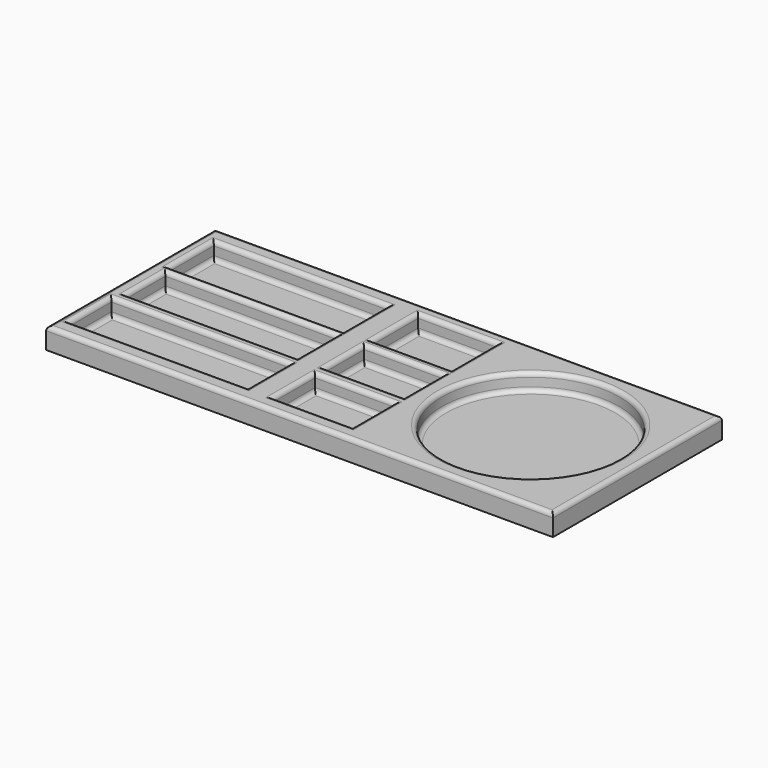
from build123d import *

# Parameters (mm, degrees)
F0_W          = 304.8
F0_H          = 127
F0_W_2        = 107.1306541562
F0_H_2        = 31.4181260765
F0_W_3        = 47.6191826165
F0_W_4        = 103.0102372169
F0_H_3        = 29.5869484544
F0_W_5        = 104.5553982258
F0_H_4        = 33.4783345461
F0_R          = 53.4565631293
F0_H_5        = 34.5084369183
F1_DEPTH      = 12.7
F2_DEPTH      = 2.54
F3_T1_DEPTH   = 104.5553982258
F3_T3_DEPTH   = 33.4783345461
F3_T5_DEPTH   = 103.0102372169
F3_T7_DEPTH   = 29.5869484544
F3_T9_DEPTH   = 107.1306541562
F3_T11_DEPTH  = 47.6191826165
F3_T13_DEPTH  = 31.4181260765
F3_T15_DEPTH  = 31.4181260765
F3_T17_DEPTH  = 34.5084369183
F3_T25_DEPTH  = 110.9053982258
F3_T29_DEPTH  = 39.8283345461
F3_T36_DEPTH  = 110.9053982258
F3_T40_DEPTH  = 39.8283345461
F3_T47_DEPTH  = 39.8283345461
F3_T51_DEPTH  = 110.9053982258
F3_T58_DEPTH  = 110.9053982258
F3_T62_DEPTH  = 39.8283345461
F3_T69_DEPTH  = 109.3602372169
F3_T73_DEPTH  = 35.9369484544
F3_T80_DEPTH  = 109.3602372169
F3_T84_DEPTH  = 35.9369484544
F3_T91_DEPTH  = 109.3602372169
F3_T95_DEPTH  = 35.9369484544
F3_T102_DEPTH = 35.9369484544
F3_T106_DEPTH = 109.3602372169
F3_T113_DEPTH = 113.4806541562
F3_T117_DEPTH = 37.7681260765
F3_T124_DEPTH = 113.4806541562
F3_T128_DEPTH = 37.7681260765
F3_T135_DEPTH = 53.9691826165
F3_T139_DEPTH = 35.9369484544
F3_T146_DEPTH = 53.9691826165
F3_T150_DEPTH = 35.9369484544
F3_T157_DEPTH = 53.9691826165
F3_T161_DEPTH = 37.7681260765
F3_T168_DEPTH = 53.9691826165
F3_T172_DEPTH = 37.7681260765
F3_T179_DEPTH = 53.9691826165
F3_T183_DEPTH = 40.8584369183
F3_T190_DEPTH = 53.9691826165
F3_T194_DEPTH = 40.8584369183
F3_T201_DEPTH = 113.4806541562
F3_T205_DEPTH = 37.7681260765
F3_T212_DEPTH = 37.7681260765
F3_T216_DEPTH = 113.4806541562
F3_T223_DEPTH = 53.9691826165
F3_T227_DEPTH = 37.7681260765
F3_T234_DEPTH = 37.7681260765
F3_T238_DEPTH = 53.9691826165
F3_T245_DEPTH = 53.9691826165
F3_T249_DEPTH = 35.9369484544
F3_T256_DEPTH = 35.9369484544
F3_T260_DEPTH = 53.9691826165
F3_T263_DEPTH = 47.6191826165
F3_T265_DEPTH = 104.5553982258
F3_T267_DEPTH = 33.4783345461
F3_T269_DEPTH = 107.1306541562
F3_T271_DEPTH = 31.4181260765
F3_T273_DEPTH = 34.5084369183
F3_T275_DEPTH = 29.5869484544
F3_T277_DEPTH = 31.4181260765
F3_T279_DEPTH = 127
F3_T281_DEPTH = 304.8
F3_T283_DEPTH = 103.0102372169
F3_T291_DEPTH = 53.9691826165
F3_T295_DEPTH = 40.8584369183
F3_T302_DEPTH = 53.9691826165
F3_T306_DEPTH = 40.8584369183
F3_T313_DEPTH = 53.9691826165
F3_T317_DEPTH = 35.9369484544
F3_T324_DEPTH = 53.9691826165
F3_T328_DEPTH = 35.9369484544
F3_T335_DEPTH = 39.8283345461
F3_T339_DEPTH = 110.9053982258
F3_T346_DEPTH = 110.9053982258
F3_T350_DEPTH = 39.8283345461
F3_T357_DEPTH = 110.9053982258
F3_T361_DEPTH = 39.8283345461
F3_T368_DEPTH = 110.9053982258
F3_T372_DEPTH = 39.8283345461
F3_T379_DEPTH = 113.4806541562
F3_T383_DEPTH = 37.7681260765
F3_T390_DEPTH = 113.4806541562
F3_T394_DEPTH = 37.7681260765
F3_T401_DEPTH = 113.4806541562
F3_T405_DEPTH = 37.7681260765
F3_T412_DEPTH = 37.7681260765
F3_T416_DEPTH = 113.4806541562
F3_T423_DEPTH = 40.8584369183
F3_T427_DEPTH = 53.9691826165
F3_T434_DEPTH = 35.9369484544
F3_T438_DEPTH = 53.9691826165
F3_T445_DEPTH = 53.9691826165
F3_T449_DEPTH = 37.7681260765
F3_T456_DEPTH = 37.7681260765
F3_T460_DEPTH = 53.9691826165
F3_T467_DEPTH = 53.9691826165
F3_T471_DEPTH = 37.7681260765
F3_T478_DEPTH = 53.9691826165
F3_T482_DEPTH = 35.9369484544
F3_T489_DEPTH = 53.9691826165
F3_T493_DEPTH = 40.8584369183
F3_T500_DEPTH = 53.9691826165
F3_T504_DEPTH = 37.7681260765
F3_T511_DEPTH = 133.35
F3_T515_DEPTH = 311.15
F3_T522_DEPTH = 133.35
F3_T526_DEPTH = 311.15
F3_T533_DEPTH = 311.15
F3_T537_DEPTH = 133.35
F3_T544_DEPTH = 311.15
F3_T548_DEPTH = 133.35
F3_T555_DEPTH = 109.3602372169
F3_T559_DEPTH = 35.9369484544
F3_T566_DEPTH = 109.3602372169
F3_T570_DEPTH = 35.9369484544
F3_T577_DEPTH = 35.9369484544
F3_T581_DEPTH = 109.3602372169
F3_T588_DEPTH = 109.3602372169
F3_T592_DEPTH = 35.9369484544


# Not quite as in the source:
# - a fillet or chamfer that OpenCascade refuses, or shapes differently, is made with other operations: its cross-section is extruded or revolved along the edge and cut away or added


with BuildPart() as f1:
    # F0 (on Top) → F1 (new body)
    with BuildSketch(Plane.XY):
        Rectangle(F0_W, F0_H)
        with Locations((-93.1070372462, -37.2266992927)):
            Rectangle(F0_W_2, F0_H_2, mode=Mode.SUBTRACT)
        with Locations((0, -37.7417504787)):
            Rectangle(F0_W_3, F0_H_2, mode=Mode.SUBTRACT)
        with Locations((-91.8194055557, 0)):
            Rectangle(F0_W_4, F0_H_3, mode=Mode.SUBTRACT)
        with Locations((-92.5919860601, 36.4256240427)):
            Rectangle(F0_W_5, F0_H_4, mode=Mode.SUBTRACT)
        Rectangle(F0_W_3, F0_H_3, mode=Mode.SUBTRACT)
        with Locations((88.1909877062, 0)):
            Circle(F0_R, mode=Mode.SUBTRACT)
        with Locations((0, 38.228303194)):
            Rectangle(F0_W_3, F0_H_5, mode=Mode.SUBTRACT)
    extrude(amount=F1_DEPTH)

    # F0 (on Top) → F2 (join)
    with BuildSketch(Plane.XY):
        with Locations((-92.5919860601, 36.4256240427)):
            Rectangle(F0_W_5, F0_H_4)
        with Locations((-91.8194055557, 0)):
            Rectangle(F0_W_4, F0_H_3)
        with Locations((-93.1070372462, -37.2266992927)):
            Rectangle(F0_W_2, F0_H_2)
        with Locations((0, -37.7417504787)):
            Rectangle(F0_W_3, F0_H_2)
        Rectangle(F0_W_3, F0_H_3)
        with Locations((0, 38.228303194)):
            Rectangle(F0_W_3, F0_H_5)
        with Locations((88.1909877062, 0)):
            Circle(F0_R)
    extrude(amount=F2_DEPTH)

    # F3: fillet of radius 2.54 on 53 edges, made by hand

    # F3_s2 → F3_t1 (join)
    with BuildSketch(Plane.YZ.offset(-144.869685173)):
        with BuildLine():
            ThreePointArc((53.1647913158, 5.08), (52.42084254, 3.2839487758), (50.6247913158, 2.54))
            Line((50.6247913158, 2.54), (50.6247913158, 2.4892))
            Line((50.6247913158, 2.4892), (53.2155913158, 2.4892))
            Line((53.2155913158, 2.4892), (53.2155913158, 5.08))
            Line((53.2155913158, 5.08), (53.1647913158, 5.08))
        make_face()
        with BuildLine():
            ThreePointArc((19.6864567697, 5.08), (20.4304055455, 3.2839487758), (22.2264567697, 2.54))
            Line((22.2264567697, 2.54), (22.2264567697, 2.4892))
            Line((22.2264567697, 2.4892), (19.6356567697, 2.4892))
            Line((19.6356567697, 2.4892), (19.6356567697, 5.08))
            Line((19.6356567697, 5.08), (19.6864567697, 5.08))
        make_face()
    extrude(amount=F3_T1_DEPTH)

    # F3_s4 → F3_t3 (join)
    with BuildSketch(Plane.XZ.offset(-53.1647913158)):
        with BuildLine():
            ThreePointArc((-40.3142869473, 5.08), (-41.058235723, 3.2839487758), (-42.8542869473, 2.54))
            Line((-42.8542869473, 2.54), (-42.8542869473, 2.4892))
            Line((-42.8542869473, 2.4892), (-40.2634869473, 2.4892))
            Line((-40.2634869473, 2.4892), (-40.2634869473, 5.08))
            Line((-40.2634869473, 5.08), (-40.3142869473, 5.08))
        make_face()
        with BuildLine():
            ThreePointArc((-144.869685173, 5.08), (-144.1257363972, 3.2839487758), (-142.329685173, 2.54))
            Line((-142.329685173, 2.54), (-142.329685173, 2.4892))
            Line((-142.329685173, 2.4892), (-144.920485173, 2.4892))
            Line((-144.920485173, 2.4892), (-144.920485173, 5.08))
            Line((-144.920485173, 5.08), (-144.869685173, 5.08))
        make_face()
    extrude(amount=F3_T3_DEPTH)

    # F3_s6 → F3_t5 (join)
    with BuildSketch(Plane.YZ.offset(-143.3245241642)):
        with BuildLine():
            ThreePointArc((14.7934742272, 5.08), (14.0495254514, 3.2839487758), (12.2534742272, 2.54))
            Line((12.2534742272, 2.54), (12.2534742272, 2.4892))
            Line((12.2534742272, 2.4892), (14.8442742272, 2.4892))
            Line((14.8442742272, 2.4892), (14.8442742272, 5.08))
            Line((14.8442742272, 5.08), (14.7934742272, 5.08))
        make_face()
        with BuildLine():
            ThreePointArc((-14.7934742272, 5.08), (-14.0495254514, 3.2839487758), (-12.2534742272, 2.54))
            Line((-12.2534742272, 2.54), (-12.2534742272, 2.4892))
            Line((-12.2534742272, 2.4892), (-14.8442742272, 2.4892))
            Line((-14.8442742272, 2.4892), (-14.8442742272, 5.08))
            Line((-14.8442742272, 5.08), (-14.7934742272, 5.08))
        make_face()
    extrude(amount=F3_T5_DEPTH)

    # F3_s8 → F3_t7 (join)
    with BuildSketch(Plane.XZ.offset(-14.7934742272)):
        with BuildLine():
            ThreePointArc((-143.3245241642, 5.08), (-142.5805753884, 3.2839487758), (-140.7845241642, 2.54))
            Line((-140.7845241642, 2.54), (-140.7845241642, 2.4892))
            Line((-140.7845241642, 2.4892), (-143.3753241642, 2.4892))
            Line((-143.3753241642, 2.4892), (-143.3753241642, 5.08))
            Line((-143.3753241642, 5.08), (-143.3245241642, 5.08))
        make_face()
        with BuildLine():
            ThreePointArc((-40.3142869473, 5.08), (-41.058235723, 3.2839487758), (-42.8542869473, 2.54))
            Line((-42.8542869473, 2.54), (-42.8542869473, 2.4892))
            Line((-42.8542869473, 2.4892), (-40.2634869473, 2.4892))
            Line((-40.2634869473, 2.4892), (-40.2634869473, 5.08))
            Line((-40.2634869473, 5.08), (-40.3142869473, 5.08))
        make_face()
        with BuildLine():
            ThreePointArc((23.8095913082, 5.08), (23.0656425324, 3.2839487758), (21.2695913082, 2.54))
            Line((21.2695913082, 2.54), (21.2695913082, 2.4892))
            Line((21.2695913082, 2.4892), (23.8603913082, 2.4892))
            Line((23.8603913082, 2.4892), (23.8603913082, 5.08))
            Line((23.8603913082, 5.08), (23.8095913082, 5.08))
        make_face()
        with BuildLine():
            ThreePointArc((-23.8095913082, 5.08), (-23.0656425324, 3.2839487758), (-21.2695913082, 2.54))
            Line((-21.2695913082, 2.54), (-21.2695913082, 2.4892))
            Line((-21.2695913082, 2.4892), (-23.8603913082, 2.4892))
            Line((-23.8603913082, 2.4892), (-23.8603913082, 5.08))
            Line((-23.8603913082, 5.08), (-23.8095913082, 5.08))
        make_face()
    extrude(amount=F3_T7_DEPTH)

    # F3_s10 → F3_t9 (join)
    with BuildSketch(Plane.YZ.offset(-146.6723643243)):
        with BuildLine():
            ThreePointArc((-21.5176362544, 5.08), (-22.2615850302, 3.2839487758), (-24.0576362544, 2.54))
            Line((-24.0576362544, 2.54), (-24.0576362544, 2.4892))
            Line((-24.0576362544, 2.4892), (-21.4668362544, 2.4892))
            Line((-21.4668362544, 2.4892), (-21.4668362544, 5.08))
            Line((-21.4668362544, 5.08), (-21.5176362544, 5.08))
        make_face()
        with BuildLine():
            ThreePointArc((-52.9357623309, 5.08), (-52.1918135551, 3.2839487758), (-50.3957623309, 2.54))
            Line((-50.3957623309, 2.54), (-50.3957623309, 2.4892))
            Line((-50.3957623309, 2.4892), (-52.9865623309, 2.4892))
            Line((-52.9865623309, 2.4892), (-52.9865623309, 5.08))
            Line((-52.9865623309, 5.08), (-52.9357623309, 5.08))
        make_face()
    extrude(amount=F3_T9_DEPTH)

    # F3_s12 → F3_t11 (join)
    with BuildSketch(Plane.YZ.offset(-23.8095913082)):
        with BuildLine():
            ThreePointArc((14.7934742272, 5.08), (14.0495254514, 3.2839487758), (12.2534742272, 2.54))
            Line((12.2534742272, 2.54), (12.2534742272, 2.4892))
            Line((12.2534742272, 2.4892), (14.8442742272, 2.4892))
            Line((14.8442742272, 2.4892), (14.8442742272, 5.08))
            Line((14.8442742272, 5.08), (14.7934742272, 5.08))
        make_face()
        with BuildLine():
            ThreePointArc((-22.0326874405, 5.08), (-22.7766362163, 3.2839487758), (-24.5726874405, 2.54))
            Line((-24.5726874405, 2.54), (-24.5726874405, 2.4892))
            Line((-24.5726874405, 2.4892), (-21.9818874405, 2.4892))
            Line((-21.9818874405, 2.4892), (-21.9818874405, 5.08))
            Line((-21.9818874405, 5.08), (-22.0326874405, 5.08))
        make_face()
        with BuildLine():
            ThreePointArc((55.4825216532, 5.08), (54.7385728774, 3.2839487758), (52.9425216532, 2.54))
            Line((52.9425216532, 2.54), (52.9425216532, 2.4892))
            Line((52.9425216532, 2.4892), (55.5333216532, 2.4892))
            Line((55.5333216532, 2.4892), (55.5333216532, 5.08))
            Line((55.5333216532, 5.08), (55.4825216532, 5.08))
        make_face()
        with BuildLine():
            ThreePointArc((-53.450813517, 5.08), (-52.7068647412, 3.2839487758), (-50.910813517, 2.54))
            Line((-50.910813517, 2.54), (-50.910813517, 2.4892))
            Line((-50.910813517, 2.4892), (-53.501613517, 2.4892))
            Line((-53.501613517, 2.4892), (-53.501613517, 5.08))
            Line((-53.501613517, 5.08), (-53.450813517, 5.08))
        make_face()
        with BuildLine():
            ThreePointArc((-14.7934742272, 5.08), (-14.0495254514, 3.2839487758), (-12.2534742272, 2.54))
            Line((-12.2534742272, 2.54), (-12.2534742272, 2.4892))
            Line((-12.2534742272, 2.4892), (-14.8442742272, 2.4892))
            Line((-14.8442742272, 2.4892), (-14.8442742272, 5.08))
            Line((-14.8442742272, 5.08), (-14.7934742272, 5.08))
        make_face()
    extrude(amount=F3_T11_DEPTH)

    # F3_s14 → F3_t13 (join)
    with BuildSketch(Plane.XZ.offset(21.5176362544)):
        with BuildLine():
            ThreePointArc((-39.5417101681, 5.08), (-40.2856589439, 3.2839487758), (-42.0817101681, 2.54))
            Line((-42.0817101681, 2.54), (-42.0817101681, 2.4892))
            Line((-42.0817101681, 2.4892), (-39.4909101681, 2.4892))
            Line((-39.4909101681, 2.4892), (-39.4909101681, 5.08))
            Line((-39.4909101681, 5.08), (-39.5417101681, 5.08))
        make_face()
        with BuildLine():
            ThreePointArc((-146.6723643243, 5.08), (-145.9284155485, 3.2839487758), (-144.1323643243, 2.54))
            Line((-144.1323643243, 2.54), (-144.1323643243, 2.4892))
            Line((-144.1323643243, 2.4892), (-146.7231643243, 2.4892))
            Line((-146.7231643243, 2.4892), (-146.7231643243, 5.08))
            Line((-146.7231643243, 5.08), (-146.6723643243, 5.08))
        make_face()
    extrude(amount=F3_T13_DEPTH)

    # F3_s16 → F3_t15 (join)
    with BuildSketch(Plane.XZ.offset(22.0326874405)):
        with BuildLine():
            ThreePointArc((23.8095913082, 5.08), (23.0656425324, 3.2839487758), (21.2695913082, 2.54))
            Line((21.2695913082, 2.54), (21.2695913082, 2.4892))
            Line((21.2695913082, 2.4892), (23.8603913082, 2.4892))
            Line((23.8603913082, 2.4892), (23.8603913082, 5.08))
            Line((23.8603913082, 5.08), (23.8095913082, 5.08))
        make_face()
        with BuildLine():
            ThreePointArc((-23.8095913082, 5.08), (-23.0656425324, 3.2839487758), (-21.2695913082, 2.54))
            Line((-21.2695913082, 2.54), (-21.2695913082, 2.4892))
            Line((-21.2695913082, 2.4892), (-23.8603913082, 2.4892))
            Line((-23.8603913082, 2.4892), (-23.8603913082, 5.08))
            Line((-23.8603913082, 5.08), (-23.8095913082, 5.08))
        make_face()
    extrude(amount=F3_T15_DEPTH)

    # F3_s18 → F3_t17 (join)
    with BuildSketch(Plane.XZ.offset(-55.4825216532)):
        with BuildLine():
            ThreePointArc((23.8095913082, 5.08), (23.0656425324, 3.2839487758), (21.2695913082, 2.54))
            Line((21.2695913082, 2.54), (21.2695913082, 2.4892))
            Line((21.2695913082, 2.4892), (23.8603913082, 2.4892))
            Line((23.8603913082, 2.4892), (23.8603913082, 5.08))
            Line((23.8603913082, 5.08), (23.8095913082, 5.08))
        make_face()
        with BuildLine():
            ThreePointArc((-23.8095913082, 5.08), (-23.0656425324, 3.2839487758), (-21.2695913082, 2.54))
            Line((-21.2695913082, 2.54), (-21.2695913082, 2.4892))
            Line((-21.2695913082, 2.4892), (-23.8603913082, 2.4892))
            Line((-23.8603913082, 2.4892), (-23.8603913082, 5.08))
            Line((-23.8603913082, 5.08), (-23.8095913082, 5.08))
        make_face()
    extrude(amount=F3_T17_DEPTH)

    # F3_s19 → F3_t20 (revolve)
    with BuildSketch(Plane.XZ):
        with BuildLine():
            ThreePointArc((141.6475508355, 5.08), (140.9036020597, 3.2839487758), (139.1075508355, 2.54))
            Line((139.1075508355, 2.54), (139.1075508355, 2.4892))
            Line((139.1075508355, 2.4892), (141.6983508355, 2.4892))
            Line((141.6983508355, 2.4892), (141.6983508355, 5.08))
            Line((141.6983508355, 5.08), (141.6475508355, 5.08))
        make_face()
    revolve(axis=Axis((88.1909877062, 0, 2.54), (0, 0, 1)))


with BuildPart() as f3_tool23:
    # F3_s24 → F3_t25 (new body)
    with BuildSketch(Plane.YZ.offset(-33.9642869473)):
        with BuildLine():
            ThreePointArc((53.1647913158, 5.08), (52.42084254, 3.2839487758), (50.6247913158, 2.54))
            Line((50.6247913158, 2.54), (50.6247913158, 2.4892))
            Line((50.6247913158, 2.4892), (53.2155913158, 2.4892))
            Line((53.2155913158, 2.4892), (53.2155913158, 5.08))
            Line((53.2155913158, 5.08), (53.1647913158, 5.08))
        make_face()
    extrude(amount=-F3_T25_DEPTH)

    split(bisect_by=Plane.YZ.offset(-40.3142869473), keep=Keep.TOP)


with BuildPart() as f3_tool27:
    # F3_s28 → F3_t29 (new body)
    with BuildSketch(Plane.XZ.offset(-19.6864567697)):
        with BuildLine():
            ThreePointArc((-40.3142869473, 5.08), (-41.058235723, 3.2839487758), (-42.8542869473, 2.54))
            Line((-42.8542869473, 2.54), (-42.8542869473, 2.4892))
            Line((-42.8542869473, 2.4892), (-40.2634869473, 2.4892))
            Line((-40.2634869473, 2.4892), (-40.2634869473, 5.08))
            Line((-40.2634869473, 5.08), (-40.3142869473, 5.08))
        make_face()
    extrude(amount=-F3_T29_DEPTH)

    split(bisect_by=Plane.XZ.offset(-53.1647913158), keep=Keep.BOTTOM)


with BuildPart() as f3_tool23_1:
    add(f3_tool23.part)

    # F3_t31: intersect F3_tool27
    add(f3_tool27.part, mode=Mode.INTERSECT)


with BuildPart() as f1_1:
    add(f1.part)

    # F3_t21: union F3_tool23
    add(f3_tool23_1.part)


with BuildPart() as f3_tool34:
    # F3_s35 → F3_t36 (new body)
    with BuildSketch(Plane.YZ.offset(-40.3142869473)):
        with BuildLine():
            ThreePointArc((53.1647913158, 5.08), (52.42084254, 3.2839487758), (50.6247913158, 2.54))
            Line((50.6247913158, 2.54), (50.6247913158, 2.4892))
            Line((50.6247913158, 2.4892), (53.2155913158, 2.4892))
            Line((53.2155913158, 2.4892), (53.2155913158, 5.08))
            Line((53.2155913158, 5.08), (53.1647913158, 5.08))
        make_face()
    extrude(amount=-F3_T36_DEPTH)

    split(bisect_by=Plane.YZ.offset(-144.869685173), keep=Keep.BOTTOM)


with BuildPart() as f3_tool38:
    # F3_s39 → F3_t40 (new body)
    with BuildSketch(Plane.XZ.offset(-59.5147913158)):
        with BuildLine():
            ThreePointArc((-144.869685173, 5.08), (-144.1257363972, 3.2839487758), (-142.329685173, 2.54))
            Line((-142.329685173, 2.54), (-142.329685173, 2.4892))
            Line((-142.329685173, 2.4892), (-144.920485173, 2.4892))
            Line((-144.920485173, 2.4892), (-144.920485173, 5.08))
            Line((-144.920485173, 5.08), (-144.869685173, 5.08))
        make_face()
    extrude(amount=F3_T40_DEPTH)

    split(bisect_by=Plane.XZ.offset(-53.1647913158), keep=Keep.BOTTOM)


with BuildPart() as f3_tool34_1:
    add(f3_tool34.part)

    # F3_t42: intersect F3_tool38
    add(f3_tool38.part, mode=Mode.INTERSECT)


with BuildPart() as f1_2:
    add(f1_1.part)

    # F3_t32: union F3_tool34
    add(f3_tool34_1.part)


with BuildPart() as f3_tool45:
    # F3_s46 → F3_t47 (new body)
    with BuildSketch(Plane.XZ.offset(-13.3364567697)):
        with BuildLine():
            ThreePointArc((-40.3142869473, 5.08), (-41.058235723, 3.2839487758), (-42.8542869473, 2.54))
            Line((-42.8542869473, 2.54), (-42.8542869473, 2.4892))
            Line((-42.8542869473, 2.4892), (-40.2634869473, 2.4892))
            Line((-40.2634869473, 2.4892), (-40.2634869473, 5.08))
            Line((-40.2634869473, 5.08), (-40.3142869473, 5.08))
        make_face()
    extrude(amount=-F3_T47_DEPTH)

    split(bisect_by=Plane.XZ.offset(-19.6864567697), keep=Keep.TOP)


with BuildPart() as f3_tool49:
    # F3_s50 → F3_t51 (new body)
    with BuildSketch(Plane.YZ.offset(-144.869685173)):
        with BuildLine():
            ThreePointArc((19.6864567697, 5.08), (20.4304055455, 3.2839487758), (22.2264567697, 2.54))
            Line((22.2264567697, 2.54), (22.2264567697, 2.4892))
            Line((22.2264567697, 2.4892), (19.6356567697, 2.4892))
            Line((19.6356567697, 2.4892), (19.6356567697, 5.08))
            Line((19.6356567697, 5.08), (19.6864567697, 5.08))
        make_face()
    extrude(amount=F3_T51_DEPTH)

    split(bisect_by=Plane.YZ.offset(-40.3142869473), keep=Keep.TOP)


with BuildPart() as f3_tool45_1:
    add(f3_tool45.part)

    # F3_t53: intersect F3_tool49
    add(f3_tool49.part, mode=Mode.INTERSECT)


with BuildPart() as f1_3:
    add(f1_2.part)

    # F3_t43: union F3_tool45
    add(f3_tool45_1.part)


with BuildPart() as f3_tool56:
    # F3_s57 → F3_t58 (new body)
    with BuildSketch(Plane.YZ.offset(-151.219685173)):
        with BuildLine():
            ThreePointArc((19.6864567697, 5.08), (20.4304055455, 3.2839487758), (22.2264567697, 2.54))
            Line((22.2264567697, 2.54), (22.2264567697, 2.4892))
            Line((22.2264567697, 2.4892), (19.6356567697, 2.4892))
            Line((19.6356567697, 2.4892), (19.6356567697, 5.08))
            Line((19.6356567697, 5.08), (19.6864567697, 5.08))
        make_face()
    extrude(amount=F3_T58_DEPTH)

    split(bisect_by=Plane.YZ.offset(-144.869685173), keep=Keep.BOTTOM)


with BuildPart() as f3_tool60:
    # F3_s61 → F3_t62 (new body)
    with BuildSketch(Plane.XZ.offset(-53.1647913158)):
        with BuildLine():
            ThreePointArc((-144.869685173, 5.08), (-144.1257363972, 3.2839487758), (-142.329685173, 2.54))
            Line((-142.329685173, 2.54), (-142.329685173, 2.4892))
            Line((-142.329685173, 2.4892), (-144.920485173, 2.4892))
            Line((-144.920485173, 2.4892), (-144.920485173, 5.08))
            Line((-144.920485173, 5.08), (-144.869685173, 5.08))
        make_face()
    extrude(amount=F3_T62_DEPTH)

    split(bisect_by=Plane.XZ.offset(-19.6864567697), keep=Keep.TOP)


with BuildPart() as f3_tool56_1:
    add(f3_tool56.part)

    # F3_t64: intersect F3_tool60
    add(f3_tool60.part, mode=Mode.INTERSECT)


with BuildPart() as f1_4:
    add(f1_3.part)

    # F3_t54: union F3_tool56
    add(f3_tool56_1.part)


with BuildPart() as f3_tool67:
    # F3_s68 → F3_t69 (new body)
    with BuildSketch(Plane.YZ.offset(-33.9642869473)):
        with BuildLine():
            ThreePointArc((14.7934742272, 5.08), (14.0495254514, 3.2839487758), (12.2534742272, 2.54))
            Line((12.2534742272, 2.54), (12.2534742272, 2.4892))
            Line((12.2534742272, 2.4892), (14.8442742272, 2.4892))
            Line((14.8442742272, 2.4892), (14.8442742272, 5.08))
            Line((14.8442742272, 5.08), (14.7934742272, 5.08))
        make_face()
    extrude(amount=-F3_T69_DEPTH)

    split(bisect_by=Plane.YZ.offset(-40.3142869473), keep=Keep.TOP)


with BuildPart() as f3_tool71:
    # F3_s72 → F3_t73 (new body)
    with BuildSketch(Plane.XZ.offset(14.7934742272)):
        with BuildLine():
            ThreePointArc((-40.3142869473, 5.08), (-41.058235723, 3.2839487758), (-42.8542869473, 2.54))
            Line((-42.8542869473, 2.54), (-42.8542869473, 2.4892))
            Line((-42.8542869473, 2.4892), (-40.2634869473, 2.4892))
            Line((-40.2634869473, 2.4892), (-40.2634869473, 5.08))
            Line((-40.2634869473, 5.08), (-40.3142869473, 5.08))
        make_face()
    extrude(amount=-F3_T73_DEPTH)

    split(bisect_by=Plane.XZ.offset(-14.7934742272), keep=Keep.BOTTOM)


with BuildPart() as f3_tool67_1:
    add(f3_tool67.part)

    # F3_t75: intersect F3_tool71
    add(f3_tool71.part, mode=Mode.INTERSECT)


with BuildPart() as f1_5:
    add(f1_4.part)

    # F3_t65: union F3_tool67
    add(f3_tool67_1.part)


with BuildPart() as f3_tool78:
    # F3_s79 → F3_t80 (new body)
    with BuildSketch(Plane.YZ.offset(-40.3142869473)):
        with BuildLine():
            ThreePointArc((14.7934742272, 5.08), (14.0495254514, 3.2839487758), (12.2534742272, 2.54))
            Line((12.2534742272, 2.54), (12.2534742272, 2.4892))
            Line((12.2534742272, 2.4892), (14.8442742272, 2.4892))
            Line((14.8442742272, 2.4892), (14.8442742272, 5.08))
            Line((14.8442742272, 5.08), (14.7934742272, 5.08))
        make_face()
    extrude(amount=-F3_T80_DEPTH)

    split(bisect_by=Plane.YZ.offset(-143.3245241642), keep=Keep.BOTTOM)


with BuildPart() as f3_tool82:
    # F3_s83 → F3_t84 (new body)
    with BuildSketch(Plane.XZ.offset(-21.1434742272)):
        with BuildLine():
            ThreePointArc((-143.3245241642, 5.08), (-142.5805753884, 3.2839487758), (-140.7845241642, 2.54))
            Line((-140.7845241642, 2.54), (-140.7845241642, 2.4892))
            Line((-140.7845241642, 2.4892), (-143.3753241642, 2.4892))
            Line((-143.3753241642, 2.4892), (-143.3753241642, 5.08))
            Line((-143.3753241642, 5.08), (-143.3245241642, 5.08))
        make_face()
    extrude(amount=F3_T84_DEPTH)

    split(bisect_by=Plane.XZ.offset(-14.7934742272), keep=Keep.BOTTOM)


with BuildPart() as f3_tool78_1:
    add(f3_tool78.part)

    # F3_t86: intersect F3_tool82
    add(f3_tool82.part, mode=Mode.INTERSECT)


with BuildPart() as f1_6:
    add(f1_5.part)

    # F3_t76: union F3_tool78
    add(f3_tool78_1.part)


with BuildPart() as f3_tool89:
    # F3_s90 → F3_t91 (new body)
    with BuildSketch(Plane.YZ.offset(-149.6745241642)):
        with BuildLine():
            ThreePointArc((-14.7934742272, 5.08), (-14.0495254514, 3.2839487758), (-12.2534742272, 2.54))
            Line((-12.2534742272, 2.54), (-12.2534742272, 2.4892))
            Line((-12.2534742272, 2.4892), (-14.8442742272, 2.4892))
            Line((-14.8442742272, 2.4892), (-14.8442742272, 5.08))
            Line((-14.8442742272, 5.08), (-14.7934742272, 5.08))
        make_face()
    extrude(amount=F3_T91_DEPTH)

    split(bisect_by=Plane.YZ.offset(-143.3245241642), keep=Keep.BOTTOM)


with BuildPart() as f3_tool93:
    # F3_s94 → F3_t95 (new body)
    with BuildSketch(Plane.XZ.offset(-14.7934742272)):
        with BuildLine():
            ThreePointArc((-143.3245241642, 5.08), (-142.5805753884, 3.2839487758), (-140.7845241642, 2.54))
            Line((-140.7845241642, 2.54), (-140.7845241642, 2.4892))
            Line((-140.7845241642, 2.4892), (-143.3753241642, 2.4892))
            Line((-143.3753241642, 2.4892), (-143.3753241642, 5.08))
            Line((-143.3753241642, 5.08), (-143.3245241642, 5.08))
        make_face()
    extrude(amount=F3_T95_DEPTH)

    split(bisect_by=Plane.XZ.offset(14.7934742272), keep=Keep.TOP)


with BuildPart() as f3_tool89_1:
    add(f3_tool89.part)

    # F3_t97: intersect F3_tool93
    add(f3_tool93.part, mode=Mode.INTERSECT)


with BuildPart() as f1_7:
    add(f1_6.part)

    # F3_t87: union F3_tool89
    add(f3_tool89_1.part)


with BuildPart() as f3_tool100:
    # F3_s101 → F3_t102 (new body)
    with BuildSketch(Plane.XZ.offset(21.1434742272)):
        with BuildLine():
            ThreePointArc((-40.3142869473, 5.08), (-41.058235723, 3.2839487758), (-42.8542869473, 2.54))
            Line((-42.8542869473, 2.54), (-42.8542869473, 2.4892))
            Line((-42.8542869473, 2.4892), (-40.2634869473, 2.4892))
            Line((-40.2634869473, 2.4892), (-40.2634869473, 5.08))
            Line((-40.2634869473, 5.08), (-40.3142869473, 5.08))
        make_face()
    extrude(amount=-F3_T102_DEPTH)

    split(bisect_by=Plane.XZ.offset(14.7934742272), keep=Keep.TOP)


with BuildPart() as f3_tool104:
    # F3_s105 → F3_t106 (new body)
    with BuildSketch(Plane.YZ.offset(-143.3245241642)):
        with BuildLine():
            ThreePointArc((-14.7934742272, 5.08), (-14.0495254514, 3.2839487758), (-12.2534742272, 2.54))
            Line((-12.2534742272, 2.54), (-12.2534742272, 2.4892))
            Line((-12.2534742272, 2.4892), (-14.8442742272, 2.4892))
            Line((-14.8442742272, 2.4892), (-14.8442742272, 5.08))
            Line((-14.8442742272, 5.08), (-14.7934742272, 5.08))
        make_face()
    extrude(amount=F3_T106_DEPTH)

    split(bisect_by=Plane.YZ.offset(-40.3142869473), keep=Keep.TOP)


with BuildPart() as f3_tool100_1:
    add(f3_tool100.part)

    # F3_t108: intersect F3_tool104
    add(f3_tool104.part, mode=Mode.INTERSECT)


with BuildPart() as f1_8:
    add(f1_7.part)

    # F3_t98: union F3_tool100
    add(f3_tool100_1.part)


with BuildPart() as f3_tool111:
    # F3_s112 → F3_t113 (new body)
    with BuildSketch(Plane.YZ.offset(-33.1917101681)):
        with BuildLine():
            ThreePointArc((-21.5176362544, 5.08), (-22.2615850302, 3.2839487758), (-24.0576362544, 2.54))
            Line((-24.0576362544, 2.54), (-24.0576362544, 2.4892))
            Line((-24.0576362544, 2.4892), (-21.4668362544, 2.4892))
            Line((-21.4668362544, 2.4892), (-21.4668362544, 5.08))
            Line((-21.4668362544, 5.08), (-21.5176362544, 5.08))
        make_face()
    extrude(amount=-F3_T113_DEPTH)

    split(bisect_by=Plane.YZ.offset(-39.5417101681), keep=Keep.TOP)


with BuildPart() as f3_tool115:
    # F3_s116 → F3_t117 (new body)
    with BuildSketch(Plane.XZ.offset(52.9357623309)):
        with BuildLine():
            ThreePointArc((-39.5417101681, 5.08), (-40.2856589439, 3.2839487758), (-42.0817101681, 2.54))
            Line((-42.0817101681, 2.54), (-42.0817101681, 2.4892))
            Line((-42.0817101681, 2.4892), (-39.4909101681, 2.4892))
            Line((-39.4909101681, 2.4892), (-39.4909101681, 5.08))
            Line((-39.4909101681, 5.08), (-39.5417101681, 5.08))
        make_face()
    extrude(amount=-F3_T117_DEPTH)

    split(bisect_by=Plane.XZ.offset(21.5176362544), keep=Keep.BOTTOM)


with BuildPart() as f3_tool111_1:
    add(f3_tool111.part)

    # F3_t119: intersect F3_tool115
    add(f3_tool115.part, mode=Mode.INTERSECT)


with BuildPart() as f1_9:
    add(f1_8.part)

    # F3_t109: union F3_tool111
    add(f3_tool111_1.part)


with BuildPart() as f3_tool122:
    # F3_s123 → F3_t124 (new body)
    with BuildSketch(Plane.YZ.offset(-39.5417101681)):
        with BuildLine():
            ThreePointArc((-21.5176362544, 5.08), (-22.2615850302, 3.2839487758), (-24.0576362544, 2.54))
            Line((-24.0576362544, 2.54), (-24.0576362544, 2.4892))
            Line((-24.0576362544, 2.4892), (-21.4668362544, 2.4892))
            Line((-21.4668362544, 2.4892), (-21.4668362544, 5.08))
            Line((-21.4668362544, 5.08), (-21.5176362544, 5.08))
        make_face()
    extrude(amount=-F3_T124_DEPTH)

    split(bisect_by=Plane.YZ.offset(-146.6723643243), keep=Keep.BOTTOM)


with BuildPart() as f3_tool126:
    # F3_s127 → F3_t128 (new body)
    with BuildSketch(Plane.XZ.offset(15.1676362544)):
        with BuildLine():
            ThreePointArc((-146.6723643243, 5.08), (-145.9284155485, 3.2839487758), (-144.1323643243, 2.54))
            Line((-144.1323643243, 2.54), (-144.1323643243, 2.4892))
            Line((-144.1323643243, 2.4892), (-146.7231643243, 2.4892))
            Line((-146.7231643243, 2.4892), (-146.7231643243, 5.08))
            Line((-146.7231643243, 5.08), (-146.6723643243, 5.08))
        make_face()
    extrude(amount=F3_T128_DEPTH)

    split(bisect_by=Plane.XZ.offset(21.5176362544), keep=Keep.BOTTOM)


with BuildPart() as f3_tool122_1:
    add(f3_tool122.part)

    # F3_t130: intersect F3_tool126
    add(f3_tool126.part, mode=Mode.INTERSECT)


with BuildPart() as f1_10:
    add(f1_9.part)

    # F3_t120: union F3_tool122
    add(f3_tool122_1.part)


with BuildPart() as f3_tool133:
    # F3_s134 → F3_t135 (new body)
    with BuildSketch(Plane.YZ.offset(30.1595913082)):
        with BuildLine():
            ThreePointArc((14.7934742272, 5.08), (14.0495254514, 3.2839487758), (12.2534742272, 2.54))
            Line((12.2534742272, 2.54), (12.2534742272, 2.4892))
            Line((12.2534742272, 2.4892), (14.8442742272, 2.4892))
            Line((14.8442742272, 2.4892), (14.8442742272, 5.08))
            Line((14.8442742272, 5.08), (14.7934742272, 5.08))
        make_face()
    extrude(amount=-F3_T135_DEPTH)

    split(bisect_by=Plane.YZ.offset(23.8095913082), keep=Keep.TOP)


with BuildPart() as f3_tool137:
    # F3_s138 → F3_t139 (new body)
    with BuildSketch(Plane.XZ.offset(14.7934742272)):
        with BuildLine():
            ThreePointArc((23.8095913082, 5.08), (23.0656425324, 3.2839487758), (21.2695913082, 2.54))
            Line((21.2695913082, 2.54), (21.2695913082, 2.4892))
            Line((21.2695913082, 2.4892), (23.8603913082, 2.4892))
            Line((23.8603913082, 2.4892), (23.8603913082, 5.08))
            Line((23.8603913082, 5.08), (23.8095913082, 5.08))
        make_face()
    extrude(amount=-F3_T139_DEPTH)

    split(bisect_by=Plane.XZ.offset(-14.7934742272), keep=Keep.BOTTOM)


with BuildPart() as f3_tool133_1:
    add(f3_tool133.part)

    # F3_t141: intersect F3_tool137
    add(f3_tool137.part, mode=Mode.INTERSECT)


with BuildPart() as f1_11:
    add(f1_10.part)

    # F3_t131: union F3_tool133
    add(f3_tool133_1.part)


with BuildPart() as f3_tool144:
    # F3_s145 → F3_t146 (new body)
    with BuildSketch(Plane.YZ.offset(23.8095913082)):
        with BuildLine():
            ThreePointArc((14.7934742272, 5.08), (14.0495254514, 3.2839487758), (12.2534742272, 2.54))
            Line((12.2534742272, 2.54), (12.2534742272, 2.4892))
            Line((12.2534742272, 2.4892), (14.8442742272, 2.4892))
            Line((14.8442742272, 2.4892), (14.8442742272, 5.08))
            Line((14.8442742272, 5.08), (14.7934742272, 5.08))
        make_face()
    extrude(amount=-F3_T146_DEPTH)

    split(bisect_by=Plane.YZ.offset(-23.8095913082), keep=Keep.BOTTOM)


with BuildPart() as f3_tool148:
    # F3_s149 → F3_t150 (new body)
    with BuildSketch(Plane.XZ.offset(-21.1434742272)):
        with BuildLine():
            ThreePointArc((-23.8095913082, 5.08), (-23.0656425324, 3.2839487758), (-21.2695913082, 2.54))
            Line((-21.2695913082, 2.54), (-21.2695913082, 2.4892))
            Line((-21.2695913082, 2.4892), (-23.8603913082, 2.4892))
            Line((-23.8603913082, 2.4892), (-23.8603913082, 5.08))
            Line((-23.8603913082, 5.08), (-23.8095913082, 5.08))
        make_face()
    extrude(amount=F3_T150_DEPTH)

    split(bisect_by=Plane.XZ.offset(-14.7934742272), keep=Keep.BOTTOM)


with BuildPart() as f3_tool144_1:
    add(f3_tool144.part)

    # F3_t152: intersect F3_tool148
    add(f3_tool148.part, mode=Mode.INTERSECT)


with BuildPart() as f1_12:
    add(f1_11.part)

    # F3_t142: union F3_tool144
    add(f3_tool144_1.part)


with BuildPart() as f3_tool155:
    # F3_s156 → F3_t157 (new body)
    with BuildSketch(Plane.YZ.offset(30.1595913082)):
        with BuildLine():
            ThreePointArc((-22.0326874405, 5.08), (-22.7766362163, 3.2839487758), (-24.5726874405, 2.54))
            Line((-24.5726874405, 2.54), (-24.5726874405, 2.4892))
            Line((-24.5726874405, 2.4892), (-21.9818874405, 2.4892))
            Line((-21.9818874405, 2.4892), (-21.9818874405, 5.08))
            Line((-21.9818874405, 5.08), (-22.0326874405, 5.08))
        make_face()
    extrude(amount=-F3_T157_DEPTH)

    split(bisect_by=Plane.YZ.offset(23.8095913082), keep=Keep.TOP)


with BuildPart() as f3_tool159:
    # F3_s160 → F3_t161 (new body)
    with BuildSketch(Plane.XZ.offset(53.450813517)):
        with BuildLine():
            ThreePointArc((23.8095913082, 5.08), (23.0656425324, 3.2839487758), (21.2695913082, 2.54))
            Line((21.2695913082, 2.54), (21.2695913082, 2.4892))
            Line((21.2695913082, 2.4892), (23.8603913082, 2.4892))
            Line((23.8603913082, 2.4892), (23.8603913082, 5.08))
            Line((23.8603913082, 5.08), (23.8095913082, 5.08))
        make_face()
    extrude(amount=-F3_T161_DEPTH)

    split(bisect_by=Plane.XZ.offset(22.0326874405), keep=Keep.BOTTOM)


with BuildPart() as f3_tool155_1:
    add(f3_tool155.part)

    # F3_t163: intersect F3_tool159
    add(f3_tool159.part, mode=Mode.INTERSECT)


with BuildPart() as f1_13:
    add(f1_12.part)

    # F3_t153: union F3_tool155
    add(f3_tool155_1.part)


with BuildPart() as f3_tool166:
    # F3_s167 → F3_t168 (new body)
    with BuildSketch(Plane.YZ.offset(23.8095913082)):
        with BuildLine():
            ThreePointArc((-22.0326874405, 5.08), (-22.7766362163, 3.2839487758), (-24.5726874405, 2.54))
            Line((-24.5726874405, 2.54), (-24.5726874405, 2.4892))
            Line((-24.5726874405, 2.4892), (-21.9818874405, 2.4892))
            Line((-21.9818874405, 2.4892), (-21.9818874405, 5.08))
            Line((-21.9818874405, 5.08), (-22.0326874405, 5.08))
        make_face()
    extrude(amount=-F3_T168_DEPTH)

    split(bisect_by=Plane.YZ.offset(-23.8095913082), keep=Keep.BOTTOM)


with BuildPart() as f3_tool170:
    # F3_s171 → F3_t172 (new body)
    with BuildSketch(Plane.XZ.offset(15.6826874405)):
        with BuildLine():
            ThreePointArc((-23.8095913082, 5.08), (-23.0656425324, 3.2839487758), (-21.2695913082, 2.54))
            Line((-21.2695913082, 2.54), (-21.2695913082, 2.4892))
            Line((-21.2695913082, 2.4892), (-23.8603913082, 2.4892))
            Line((-23.8603913082, 2.4892), (-23.8603913082, 5.08))
            Line((-23.8603913082, 5.08), (-23.8095913082, 5.08))
        make_face()
    extrude(amount=F3_T172_DEPTH)

    split(bisect_by=Plane.XZ.offset(22.0326874405), keep=Keep.BOTTOM)


with BuildPart() as f3_tool166_1:
    add(f3_tool166.part)

    # F3_t174: intersect F3_tool170
    add(f3_tool170.part, mode=Mode.INTERSECT)


with BuildPart() as f1_14:
    add(f1_13.part)

    # F3_t164: union F3_tool166
    add(f3_tool166_1.part)


with BuildPart() as f3_tool177:
    # F3_s178 → F3_t179 (new body)
    with BuildSketch(Plane.YZ.offset(30.1595913082)):
        with BuildLine():
            ThreePointArc((55.4825216532, 5.08), (54.7385728774, 3.2839487758), (52.9425216532, 2.54))
            Line((52.9425216532, 2.54), (52.9425216532, 2.4892))
            Line((52.9425216532, 2.4892), (55.5333216532, 2.4892))
            Line((55.5333216532, 2.4892), (55.5333216532, 5.08))
            Line((55.5333216532, 5.08), (55.4825216532, 5.08))
        make_face()
    extrude(amount=-F3_T179_DEPTH)

    split(bisect_by=Plane.YZ.offset(23.8095913082), keep=Keep.TOP)


with BuildPart() as f3_tool181:
    # F3_s182 → F3_t183 (new body)
    with BuildSketch(Plane.XZ.offset(-20.9740847349)):
        with BuildLine():
            ThreePointArc((23.8095913082, 5.08), (23.0656425324, 3.2839487758), (21.2695913082, 2.54))
            Line((21.2695913082, 2.54), (21.2695913082, 2.4892))
            Line((21.2695913082, 2.4892), (23.8603913082, 2.4892))
            Line((23.8603913082, 2.4892), (23.8603913082, 5.08))
            Line((23.8603913082, 5.08), (23.8095913082, 5.08))
        make_face()
    extrude(amount=-F3_T183_DEPTH)

    split(bisect_by=Plane.XZ.offset(-55.4825216532), keep=Keep.BOTTOM)


with BuildPart() as f3_tool177_1:
    add(f3_tool177.part)

    # F3_t185: intersect F3_tool181
    add(f3_tool181.part, mode=Mode.INTERSECT)


with BuildPart() as f1_15:
    add(f1_14.part)

    # F3_t175: union F3_tool177
    add(f3_tool177_1.part)


with BuildPart() as f3_tool188:
    # F3_s189 → F3_t190 (new body)
    with BuildSketch(Plane.YZ.offset(23.8095913082)):
        with BuildLine():
            ThreePointArc((55.4825216532, 5.08), (54.7385728774, 3.2839487758), (52.9425216532, 2.54))
            Line((52.9425216532, 2.54), (52.9425216532, 2.4892))
            Line((52.9425216532, 2.4892), (55.5333216532, 2.4892))
            Line((55.5333216532, 2.4892), (55.5333216532, 5.08))
            Line((55.5333216532, 5.08), (55.4825216532, 5.08))
        make_face()
    extrude(amount=-F3_T190_DEPTH)

    split(bisect_by=Plane.YZ.offset(-23.8095913082), keep=Keep.BOTTOM)


with BuildPart() as f3_tool192:
    # F3_s193 → F3_t194 (new body)
    with BuildSketch(Plane.XZ.offset(-61.8325216532)):
        with BuildLine():
            ThreePointArc((-23.8095913082, 5.08), (-23.0656425324, 3.2839487758), (-21.2695913082, 2.54))
            Line((-21.2695913082, 2.54), (-21.2695913082, 2.4892))
            Line((-21.2695913082, 2.4892), (-23.8603913082, 2.4892))
            Line((-23.8603913082, 2.4892), (-23.8603913082, 5.08))
            Line((-23.8603913082, 5.08), (-23.8095913082, 5.08))
        make_face()
    extrude(amount=F3_T194_DEPTH)

    split(bisect_by=Plane.XZ.offset(-55.4825216532), keep=Keep.BOTTOM)


with BuildPart() as f3_tool188_1:
    add(f3_tool188.part)

    # F3_t196: intersect F3_tool192
    add(f3_tool192.part, mode=Mode.INTERSECT)


with BuildPart() as f1_16:
    add(f1_15.part)

    # F3_t186: union F3_tool188
    add(f3_tool188_1.part)


with BuildPart() as f3_tool199:
    # F3_s200 → F3_t201 (new body)
    with BuildSketch(Plane.YZ.offset(-153.0223643243)):
        with BuildLine():
            ThreePointArc((-52.9357623309, 5.08), (-52.1918135551, 3.2839487758), (-50.3957623309, 2.54))
            Line((-50.3957623309, 2.54), (-50.3957623309, 2.4892))
            Line((-50.3957623309, 2.4892), (-52.9865623309, 2.4892))
            Line((-52.9865623309, 2.4892), (-52.9865623309, 5.08))
            Line((-52.9865623309, 5.08), (-52.9357623309, 5.08))
        make_face()
    extrude(amount=F3_T201_DEPTH)

    split(bisect_by=Plane.YZ.offset(-146.6723643243), keep=Keep.BOTTOM)


with BuildPart() as f3_tool203:
    # F3_s204 → F3_t205 (new body)
    with BuildSketch(Plane.XZ.offset(21.5176362544)):
        with BuildLine():
            ThreePointArc((-146.6723643243, 5.08), (-145.9284155485, 3.2839487758), (-144.1323643243, 2.54))
            Line((-144.1323643243, 2.54), (-144.1323643243, 2.4892))
            Line((-144.1323643243, 2.4892), (-146.7231643243, 2.4892))
            Line((-146.7231643243, 2.4892), (-146.7231643243, 5.08))
            Line((-146.7231643243, 5.08), (-146.6723643243, 5.08))
        make_face()
    extrude(amount=F3_T205_DEPTH)

    split(bisect_by=Plane.XZ.offset(52.9357623309), keep=Keep.TOP)


with BuildPart() as f3_tool199_1:
    add(f3_tool199.part)

    # F3_t207: intersect F3_tool203
    add(f3_tool203.part, mode=Mode.INTERSECT)


with BuildPart() as f1_17:
    add(f1_16.part)

    # F3_t197: union F3_tool199
    add(f3_tool199_1.part)


with BuildPart() as f3_tool210:
    # F3_s211 → F3_t212 (new body)
    with BuildSketch(Plane.XZ.offset(59.2857623309)):
        with BuildLine():
            ThreePointArc((-39.5417101681, 5.08), (-40.2856589439, 3.2839487758), (-42.0817101681, 2.54))
            Line((-42.0817101681, 2.54), (-42.0817101681, 2.4892))
            Line((-42.0817101681, 2.4892), (-39.4909101681, 2.4892))
            Line((-39.4909101681, 2.4892), (-39.4909101681, 5.08))
            Line((-39.4909101681, 5.08), (-39.5417101681, 5.08))
        make_face()
    extrude(amount=-F3_T212_DEPTH)

    split(bisect_by=Plane.XZ.offset(52.9357623309), keep=Keep.TOP)


with BuildPart() as f3_tool214:
    # F3_s215 → F3_t216 (new body)
    with BuildSketch(Plane.YZ.offset(-146.6723643243)):
        with BuildLine():
            ThreePointArc((-52.9357623309, 5.08), (-52.1918135551, 3.2839487758), (-50.3957623309, 2.54))
            Line((-50.3957623309, 2.54), (-50.3957623309, 2.4892))
            Line((-50.3957623309, 2.4892), (-52.9865623309, 2.4892))
            Line((-52.9865623309, 2.4892), (-52.9865623309, 5.08))
            Line((-52.9865623309, 5.08), (-52.9357623309, 5.08))
        make_face()
    extrude(amount=F3_T216_DEPTH)

    split(bisect_by=Plane.YZ.offset(-39.5417101681), keep=Keep.TOP)


with BuildPart() as f3_tool210_1:
    add(f3_tool210.part)

    # F3_t218: intersect F3_tool214
    add(f3_tool214.part, mode=Mode.INTERSECT)


with BuildPart() as f1_18:
    add(f1_17.part)

    # F3_t208: union F3_tool210
    add(f3_tool210_1.part)


with BuildPart() as f3_tool221:
    # F3_s222 → F3_t223 (new body)
    with BuildSketch(Plane.YZ.offset(-30.1595913082)):
        with BuildLine():
            ThreePointArc((-53.450813517, 5.08), (-52.7068647412, 3.2839487758), (-50.910813517, 2.54))
            Line((-50.910813517, 2.54), (-50.910813517, 2.4892))
            Line((-50.910813517, 2.4892), (-53.501613517, 2.4892))
            Line((-53.501613517, 2.4892), (-53.501613517, 5.08))
            Line((-53.501613517, 5.08), (-53.450813517, 5.08))
        make_face()
    extrude(amount=F3_T223_DEPTH)

    split(bisect_by=Plane.YZ.offset(-23.8095913082), keep=Keep.BOTTOM)


with BuildPart() as f3_tool225:
    # F3_s226 → F3_t227 (new body)
    with BuildSketch(Plane.XZ.offset(22.0326874405)):
        with BuildLine():
            ThreePointArc((-23.8095913082, 5.08), (-23.0656425324, 3.2839487758), (-21.2695913082, 2.54))
            Line((-21.2695913082, 2.54), (-21.2695913082, 2.4892))
            Line((-21.2695913082, 2.4892), (-23.8603913082, 2.4892))
            Line((-23.8603913082, 2.4892), (-23.8603913082, 5.08))
            Line((-23.8603913082, 5.08), (-23.8095913082, 5.08))
        make_face()
    extrude(amount=F3_T227_DEPTH)

    split(bisect_by=Plane.XZ.offset(53.450813517), keep=Keep.TOP)


with BuildPart() as f3_tool221_1:
    add(f3_tool221.part)

    # F3_t229: intersect F3_tool225
    add(f3_tool225.part, mode=Mode.INTERSECT)


with BuildPart() as f1_19:
    add(f1_18.part)

    # F3_t219: union F3_tool221
    add(f3_tool221_1.part)


with BuildPart() as f3_tool232:
    # F3_s233 → F3_t234 (new body)
    with BuildSketch(Plane.XZ.offset(59.800813517)):
        with BuildLine():
            ThreePointArc((23.8095913082, 5.08), (23.0656425324, 3.2839487758), (21.2695913082, 2.54))
            Line((21.2695913082, 2.54), (21.2695913082, 2.4892))
            Line((21.2695913082, 2.4892), (23.8603913082, 2.4892))
            Line((23.8603913082, 2.4892), (23.8603913082, 5.08))
            Line((23.8603913082, 5.08), (23.8095913082, 5.08))
        make_face()
    extrude(amount=-F3_T234_DEPTH)

    split(bisect_by=Plane.XZ.offset(53.450813517), keep=Keep.TOP)


with BuildPart() as f3_tool236:
    # F3_s237 → F3_t238 (new body)
    with BuildSketch(Plane.YZ.offset(-23.8095913082)):
        with BuildLine():
            ThreePointArc((-53.450813517, 5.08), (-52.7068647412, 3.2839487758), (-50.910813517, 2.54))
            Line((-50.910813517, 2.54), (-50.910813517, 2.4892))
            Line((-50.910813517, 2.4892), (-53.501613517, 2.4892))
            Line((-53.501613517, 2.4892), (-53.501613517, 5.08))
            Line((-53.501613517, 5.08), (-53.450813517, 5.08))
        make_face()
    extrude(amount=F3_T238_DEPTH)

    split(bisect_by=Plane.YZ.offset(23.8095913082), keep=Keep.TOP)


with BuildPart() as f3_tool232_1:
    add(f3_tool232.part)

    # F3_t240: intersect F3_tool236
    add(f3_tool236.part, mode=Mode.INTERSECT)


with BuildPart() as f1_20:
    add(f1_19.part)

    # F3_t230: union F3_tool232
    add(f3_tool232_1.part)


with BuildPart() as f3_tool243:
    # F3_s244 → F3_t245 (new body)
    with BuildSketch(Plane.YZ.offset(-30.1595913082)):
        with BuildLine():
            ThreePointArc((-14.7934742272, 5.08), (-14.0495254514, 3.2839487758), (-12.2534742272, 2.54))
            Line((-12.2534742272, 2.54), (-12.2534742272, 2.4892))
            Line((-12.2534742272, 2.4892), (-14.8442742272, 2.4892))
            Line((-14.8442742272, 2.4892), (-14.8442742272, 5.08))
            Line((-14.8442742272, 5.08), (-14.7934742272, 5.08))
        make_face()
    extrude(amount=F3_T245_DEPTH)

    split(bisect_by=Plane.YZ.offset(-23.8095913082), keep=Keep.BOTTOM)


with BuildPart() as f3_tool247:
    # F3_s248 → F3_t249 (new body)
    with BuildSketch(Plane.XZ.offset(-14.7934742272)):
        with BuildLine():
            ThreePointArc((-23.8095913082, 5.08), (-23.0656425324, 3.2839487758), (-21.2695913082, 2.54))
            Line((-21.2695913082, 2.54), (-21.2695913082, 2.4892))
            Line((-21.2695913082, 2.4892), (-23.8603913082, 2.4892))
            Line((-23.8603913082, 2.4892), (-23.8603913082, 5.08))
            Line((-23.8603913082, 5.08), (-23.8095913082, 5.08))
        make_face()
    extrude(amount=F3_T249_DEPTH)

    split(bisect_by=Plane.XZ.offset(14.7934742272), keep=Keep.TOP)


with BuildPart() as f3_tool243_1:
    add(f3_tool243.part)

    # F3_t251: intersect F3_tool247
    add(f3_tool247.part, mode=Mode.INTERSECT)


with BuildPart() as f1_21:
    add(f1_20.part)

    # F3_t241: union F3_tool243
    add(f3_tool243_1.part)


with BuildPart() as f3_tool254:
    # F3_s255 → F3_t256 (new body)
    with BuildSketch(Plane.XZ.offset(21.1434742272)):
        with BuildLine():
            ThreePointArc((23.8095913082, 5.08), (23.0656425324, 3.2839487758), (21.2695913082, 2.54))
            Line((21.2695913082, 2.54), (21.2695913082, 2.4892))
            Line((21.2695913082, 2.4892), (23.8603913082, 2.4892))
            Line((23.8603913082, 2.4892), (23.8603913082, 5.08))
            Line((23.8603913082, 5.08), (23.8095913082, 5.08))
        make_face()
    extrude(amount=-F3_T256_DEPTH)

    split(bisect_by=Plane.XZ.offset(14.7934742272), keep=Keep.TOP)


with BuildPart() as f3_tool258:
    # F3_s259 → F3_t260 (new body)
    with BuildSketch(Plane.YZ.offset(-23.8095913082)):
        with BuildLine():
            ThreePointArc((-14.7934742272, 5.08), (-14.0495254514, 3.2839487758), (-12.2534742272, 2.54))
            Line((-12.2534742272, 2.54), (-12.2534742272, 2.4892))
            Line((-12.2534742272, 2.4892), (-14.8442742272, 2.4892))
            Line((-14.8442742272, 2.4892), (-14.8442742272, 5.08))
            Line((-14.8442742272, 5.08), (-14.7934742272, 5.08))
        make_face()
    extrude(amount=F3_T260_DEPTH)

    split(bisect_by=Plane.YZ.offset(23.8095913082), keep=Keep.TOP)


with BuildPart() as f3_tool254_1:
    add(f3_tool254.part)

    # F3_t262: intersect F3_tool258
    add(f3_tool258.part, mode=Mode.INTERSECT)


with BuildPart() as f1_22:
    add(f1_21.part)

    # F3_t252: union F3_tool254
    add(f3_tool254_1.part)

    # F3_s264 → F3_t263 (cut)
    with BuildSketch(Plane.YZ.offset(-23.8095913082)):
        with BuildLine():
            ThreePointArc((58.0225216532, 12.7), (56.226470429, 11.9560512242), (55.4825216532, 10.16))
            Line((55.4825216532, 10.16), (55.4317216532, 10.16))
            Line((55.4317216532, 10.16), (55.4317216532, 12.7508))
            Line((55.4317216532, 12.7508), (58.0225216532, 12.7508))
            Line((58.0225216532, 12.7508), (58.0225216532, 12.7))
        make_face()
        with BuildLine():
            ThreePointArc((17.3334742272, 12.7), (15.537423003, 11.9560512242), (14.7934742272, 10.16))
            Line((14.7934742272, 10.16), (14.7426742272, 10.16))
            Line((14.7426742272, 10.16), (14.7426742272, 12.7508))
            Line((14.7426742272, 12.7508), (17.3334742272, 12.7508))
            Line((17.3334742272, 12.7508), (17.3334742272, 12.7))
        make_face()
        with BuildLine():
            ThreePointArc((-19.4926874405, 12.7), (-21.2887386647, 11.9560512242), (-22.0326874405, 10.16))
            Line((-22.0326874405, 10.16), (-22.0834874405, 10.16))
            Line((-22.0834874405, 10.16), (-22.0834874405, 12.7508))
            Line((-22.0834874405, 12.7508), (-19.4926874405, 12.7508))
            Line((-19.4926874405, 12.7508), (-19.4926874405, 12.7))
        make_face()
        with BuildLine():
            ThreePointArc((-17.3334742272, 12.7), (-15.537423003, 11.9560512242), (-14.7934742272, 10.16))
            Line((-14.7934742272, 10.16), (-14.7426742272, 10.16))
            Line((-14.7426742272, 10.16), (-14.7426742272, 12.7508))
            Line((-14.7426742272, 12.7508), (-17.3334742272, 12.7508))
            Line((-17.3334742272, 12.7508), (-17.3334742272, 12.7))
        make_face()
        with BuildLine():
            ThreePointArc((18.4340847349, 12.7), (20.2301359591, 11.9560512242), (20.9740847349, 10.16))
            Line((20.9740847349, 10.16), (21.0248847349, 10.16))
            Line((21.0248847349, 10.16), (21.0248847349, 12.7508))
            Line((21.0248847349, 12.7508), (18.4340847349, 12.7508))
            Line((18.4340847349, 12.7508), (18.4340847349, 12.7))
        make_face()
        with BuildLine():
            ThreePointArc((-55.990813517, 12.7), (-54.1947622928, 11.9560512242), (-53.450813517, 10.16))
            Line((-53.450813517, 10.16), (-53.400013517, 10.16))
            Line((-53.400013517, 10.16), (-53.400013517, 12.7508))
            Line((-53.400013517, 12.7508), (-55.990813517, 12.7508))
            Line((-55.990813517, 12.7508), (-55.990813517, 12.7))
        make_face()
    extrude(amount=F3_T263_DEPTH, mode=Mode.SUBTRACT)

    # F3_s266 → F3_t265 (cut)
    with BuildSketch(Plane.YZ.offset(-144.869685173)):
        with BuildLine():
            ThreePointArc((17.1464567697, 12.7), (18.9425079939, 11.9560512242), (19.6864567697, 10.16))
            Line((19.6864567697, 10.16), (19.7372567697, 10.16))
            Line((19.7372567697, 10.16), (19.7372567697, 12.7508))
            Line((19.7372567697, 12.7508), (17.1464567697, 12.7508))
            Line((17.1464567697, 12.7508), (17.1464567697, 12.7))
        make_face()
        with BuildLine():
            ThreePointArc((55.7047913158, 12.7), (53.9087400916, 11.9560512242), (53.1647913158, 10.16))
            Line((53.1647913158, 10.16), (53.1139913158, 10.16))
            Line((53.1139913158, 10.16), (53.1139913158, 12.7508))
            Line((53.1139913158, 12.7508), (55.7047913158, 12.7508))
            Line((55.7047913158, 12.7508), (55.7047913158, 12.7))
        make_face()
    extrude(amount=F3_T265_DEPTH, mode=Mode.SUBTRACT)

    # F3_s268 → F3_t267 (cut)
    with BuildSketch(Plane.XZ.offset(-53.1647913158)):
        with BuildLine():
            ThreePointArc((-37.7742869473, 12.7), (-39.5703381715, 11.9560512242), (-40.3142869473, 10.16))
            Line((-40.3142869473, 10.16), (-40.3650869473, 10.16))
            Line((-40.3650869473, 10.16), (-40.3650869473, 12.7508))
            Line((-40.3650869473, 12.7508), (-37.7742869473, 12.7508))
            Line((-37.7742869473, 12.7508), (-37.7742869473, 12.7))
        make_face()
        with BuildLine():
            ThreePointArc((-147.409685173, 12.7), (-145.6136339488, 11.9560512242), (-144.869685173, 10.16))
            Line((-144.869685173, 10.16), (-144.818885173, 10.16))
            Line((-144.818885173, 10.16), (-144.818885173, 12.7508))
            Line((-144.818885173, 12.7508), (-147.409685173, 12.7508))
            Line((-147.409685173, 12.7508), (-147.409685173, 12.7))
        make_face()
    extrude(amount=F3_T267_DEPTH, mode=Mode.SUBTRACT)

    # F3_s270 → F3_t269 (cut)
    with BuildSketch(Plane.YZ.offset(-146.6723643243)):
        with BuildLine():
            ThreePointArc((-18.9776362544, 12.7), (-20.7736874786, 11.9560512242), (-21.5176362544, 10.16))
            Line((-21.5176362544, 10.16), (-21.5684362544, 10.16))
            Line((-21.5684362544, 10.16), (-21.5684362544, 12.7508))
            Line((-21.5684362544, 12.7508), (-18.9776362544, 12.7508))
            Line((-18.9776362544, 12.7508), (-18.9776362544, 12.7))
        make_face()
        with BuildLine():
            ThreePointArc((-55.4757623309, 12.7), (-53.6797111067, 11.9560512242), (-52.9357623309, 10.16))
            Line((-52.9357623309, 10.16), (-52.8849623309, 10.16))
            Line((-52.8849623309, 10.16), (-52.8849623309, 12.7508))
            Line((-52.8849623309, 12.7508), (-55.4757623309, 12.7508))
            Line((-55.4757623309, 12.7508), (-55.4757623309, 12.7))
        make_face()
    extrude(amount=F3_T269_DEPTH, mode=Mode.SUBTRACT)

    # F3_s272 → F3_t271 (cut)
    with BuildSketch(Plane.XZ.offset(21.5176362544)):
        with BuildLine():
            ThreePointArc((-149.2123643243, 12.7), (-147.4163131001, 11.9560512242), (-146.6723643243, 10.16))
            Line((-146.6723643243, 10.16), (-146.6215643243, 10.16))
            Line((-146.6215643243, 10.16), (-146.6215643243, 12.7508))
            Line((-146.6215643243, 12.7508), (-149.2123643243, 12.7508))
            Line((-149.2123643243, 12.7508), (-149.2123643243, 12.7))
        make_face()
        with BuildLine():
            ThreePointArc((-37.0017101681, 12.7), (-38.7977613923, 11.9560512242), (-39.5417101681, 10.16))
            Line((-39.5417101681, 10.16), (-39.5925101681, 10.16))
            Line((-39.5925101681, 10.16), (-39.5925101681, 12.7508))
            Line((-39.5925101681, 12.7508), (-37.0017101681, 12.7508))
            Line((-37.0017101681, 12.7508), (-37.0017101681, 12.7))
        make_face()
    extrude(amount=F3_T271_DEPTH, mode=Mode.SUBTRACT)

    # F3_s274 → F3_t273 (cut)
    with BuildSketch(Plane.XZ.offset(-55.4825216532)):
        with BuildLine():
            ThreePointArc((26.3495913082, 12.7), (24.553540084, 11.9560512242), (23.8095913082, 10.16))
            Line((23.8095913082, 10.16), (23.7587913082, 10.16))
            Line((23.7587913082, 10.16), (23.7587913082, 12.7508))
            Line((23.7587913082, 12.7508), (26.3495913082, 12.7508))
            Line((26.3495913082, 12.7508), (26.3495913082, 12.7))
        make_face()
        with BuildLine():
            ThreePointArc((-26.3495913082, 12.7), (-24.553540084, 11.9560512242), (-23.8095913082, 10.16))
            Line((-23.8095913082, 10.16), (-23.7587913082, 10.16))
            Line((-23.7587913082, 10.16), (-23.7587913082, 12.7508))
            Line((-23.7587913082, 12.7508), (-26.3495913082, 12.7508))
            Line((-26.3495913082, 12.7508), (-26.3495913082, 12.7))
        make_face()
    extrude(amount=F3_T273_DEPTH, mode=Mode.SUBTRACT)

    # F3_s276 → F3_t275 (cut)
    with BuildSketch(Plane.XZ.offset(-14.7934742272)):
        with BuildLine():
            ThreePointArc((26.3495913082, 12.7), (24.553540084, 11.9560512242), (23.8095913082, 10.16))
            Line((23.8095913082, 10.16), (23.7587913082, 10.16))
            Line((23.7587913082, 10.16), (23.7587913082, 12.7508))
            Line((23.7587913082, 12.7508), (26.3495913082, 12.7508))
            Line((26.3495913082, 12.7508), (26.3495913082, 12.7))
        make_face()
        with BuildLine():
            ThreePointArc((-37.7742869473, 12.7), (-39.5703381715, 11.9560512242), (-40.3142869473, 10.16))
            Line((-40.3142869473, 10.16), (-40.3650869473, 10.16))
            Line((-40.3650869473, 10.16), (-40.3650869473, 12.7508))
            Line((-40.3650869473, 12.7508), (-37.7742869473, 12.7508))
            Line((-37.7742869473, 12.7508), (-37.7742869473, 12.7))
        make_face()
        with BuildLine():
            ThreePointArc((-145.8645241642, 12.7), (-144.06847294, 11.9560512242), (-143.3245241642, 10.16))
            Line((-143.3245241642, 10.16), (-143.2737241642, 10.16))
            Line((-143.2737241642, 10.16), (-143.2737241642, 12.7508))
            Line((-143.2737241642, 12.7508), (-145.8645241642, 12.7508))
            Line((-145.8645241642, 12.7508), (-145.8645241642, 12.7))
        make_face()
        with BuildLine():
            ThreePointArc((-26.3495913082, 12.7), (-24.553540084, 11.9560512242), (-23.8095913082, 10.16))
            Line((-23.8095913082, 10.16), (-23.7587913082, 10.16))
            Line((-23.7587913082, 10.16), (-23.7587913082, 12.7508))
            Line((-23.7587913082, 12.7508), (-26.3495913082, 12.7508))
            Line((-26.3495913082, 12.7508), (-26.3495913082, 12.7))
        make_face()
    extrude(amount=F3_T275_DEPTH, mode=Mode.SUBTRACT)

    # F3_s278 → F3_t277 (cut)
    with BuildSketch(Plane.XZ.offset(22.0326874405)):
        with BuildLine():
            ThreePointArc((26.3495913082, 12.7), (24.553540084, 11.9560512242), (23.8095913082, 10.16))
            Line((23.8095913082, 10.16), (23.7587913082, 10.16))
            Line((23.7587913082, 10.16), (23.7587913082, 12.7508))
            Line((23.7587913082, 12.7508), (26.3495913082, 12.7508))
            Line((26.3495913082, 12.7508), (26.3495913082, 12.7))
        make_face()
        with BuildLine():
            ThreePointArc((-26.3495913082, 12.7), (-24.553540084, 11.9560512242), (-23.8095913082, 10.16))
            Line((-23.8095913082, 10.16), (-23.7587913082, 10.16))
            Line((-23.7587913082, 10.16), (-23.7587913082, 12.7508))
            Line((-23.7587913082, 12.7508), (-26.3495913082, 12.7508))
            Line((-26.3495913082, 12.7508), (-26.3495913082, 12.7))
        make_face()
    extrude(amount=F3_T277_DEPTH, mode=Mode.SUBTRACT)

    # F3_s280 → F3_t279 (cut)
    with BuildSketch(Plane.XZ.offset(-63.5)):
        with BuildLine():
            ThreePointArc((152.4, 10.16), (151.6560512242, 11.9560512242), (149.86, 12.7))
            Line((149.86, 12.7), (149.86, 12.7508))
            Line((149.86, 12.7508), (152.4508, 12.7508))
            Line((152.4508, 12.7508), (152.4508, 10.16))
            Line((152.4508, 10.16), (152.4, 10.16))
        make_face()
        with BuildLine():
            ThreePointArc((-149.86, 12.7), (-151.6560512242, 11.9560512242), (-152.4, 10.16))
            Line((-152.4, 10.16), (-152.4508, 10.16))
            Line((-152.4508, 10.16), (-152.4508, 12.7508))
            Line((-152.4508, 12.7508), (-149.86, 12.7508))
            Line((-149.86, 12.7508), (-149.86, 12.7))
        make_face()
    extrude(amount=F3_T279_DEPTH, mode=Mode.SUBTRACT)

    # F3_s282 → F3_t281 (cut)
    with BuildSketch(Plane.YZ.offset(-152.4)):
        with BuildLine():
            ThreePointArc((63.5, 10.16), (62.7560512242, 11.9560512242), (60.96, 12.7))
            Line((60.96, 12.7), (60.96, 12.7508))
            Line((60.96, 12.7508), (63.5508, 12.7508))
            Line((63.5508, 12.7508), (63.5508, 10.16))
            Line((63.5508, 10.16), (63.5, 10.16))
        make_face()
        with BuildLine():
            ThreePointArc((-63.5, 10.16), (-62.7560512242, 11.9560512242), (-60.96, 12.7))
            Line((-60.96, 12.7), (-60.96, 12.7508))
            Line((-60.96, 12.7508), (-63.5508, 12.7508))
            Line((-63.5508, 12.7508), (-63.5508, 10.16))
            Line((-63.5508, 10.16), (-63.5, 10.16))
        make_face()
    extrude(amount=F3_T281_DEPTH, mode=Mode.SUBTRACT)

    # F3_s284 → F3_t283 (cut)
    with BuildSketch(Plane.YZ.offset(-143.3245241642)):
        with BuildLine():
            ThreePointArc((17.3334742272, 12.7), (15.537423003, 11.9560512242), (14.7934742272, 10.16))
            Line((14.7934742272, 10.16), (14.7426742272, 10.16))
            Line((14.7426742272, 10.16), (14.7426742272, 12.7508))
            Line((14.7426742272, 12.7508), (17.3334742272, 12.7508))
            Line((17.3334742272, 12.7508), (17.3334742272, 12.7))
        make_face()
        with BuildLine():
            ThreePointArc((-17.3334742272, 12.7), (-15.537423003, 11.9560512242), (-14.7934742272, 10.16))
            Line((-14.7934742272, 10.16), (-14.7426742272, 10.16))
            Line((-14.7426742272, 10.16), (-14.7426742272, 12.7508))
            Line((-14.7426742272, 12.7508), (-17.3334742272, 12.7508))
            Line((-17.3334742272, 12.7508), (-17.3334742272, 12.7))
        make_face()
    extrude(amount=F3_T283_DEPTH, mode=Mode.SUBTRACT)

    # F3_s285 → F3_t286 (revolve, cut)
    with BuildSketch(Plane.XZ):
        with BuildLine():
            ThreePointArc((144.1875508355, 12.7), (142.3914996113, 11.9560512242), (141.6475508355, 10.16))
            Line((141.6475508355, 10.16), (141.5967508355, 10.16))
            Line((141.5967508355, 10.16), (141.5967508355, 12.7508))
            Line((141.5967508355, 12.7508), (144.1875508355, 12.7508))
            Line((144.1875508355, 12.7508), (144.1875508355, 12.7))
        make_face()
    revolve(axis=Axis((88.1909877062, 0, 12.7), (0, 0, 1)), mode=Mode.SUBTRACT)


with BuildPart() as f3_tool289:
    # F3_s290 → F3_t291 (new body)
    with BuildSketch(Plane.YZ.offset(-30.1595913082)):
        with BuildLine():
            ThreePointArc((58.0225216532, 12.7), (56.226470429, 11.9560512242), (55.4825216532, 10.16))
            Line((55.4825216532, 10.16), (55.4317216532, 10.16))
            Line((55.4317216532, 10.16), (55.4317216532, 12.7508))
            Line((55.4317216532, 12.7508), (58.0225216532, 12.7508))
            Line((58.0225216532, 12.7508), (58.0225216532, 12.7))
        make_face()
    extrude(amount=F3_T291_DEPTH)

    split(bisect_by=Plane.YZ.offset(-23.8095913082), keep=Keep.BOTTOM)


with BuildPart() as f3_tool293:
    # F3_s294 → F3_t295 (new body)
    with BuildSketch(Plane.XZ.offset(-20.9740847349)):
        with BuildLine():
            ThreePointArc((-26.3495913082, 12.7), (-24.553540084, 11.9560512242), (-23.8095913082, 10.16))
            Line((-23.8095913082, 10.16), (-23.7587913082, 10.16))
            Line((-23.7587913082, 10.16), (-23.7587913082, 12.7508))
            Line((-23.7587913082, 12.7508), (-26.3495913082, 12.7508))
            Line((-26.3495913082, 12.7508), (-26.3495913082, 12.7))
        make_face()
    extrude(amount=-F3_T295_DEPTH)

    split(bisect_by=Plane.XZ.offset(-55.4825216532), keep=Keep.BOTTOM)


with BuildPart() as f3_tool289_1:
    add(f3_tool289.part)

    # F3_t297: intersect F3_tool293
    add(f3_tool293.part, mode=Mode.INTERSECT)


with BuildPart() as f1_23:
    add(f1_22.part)

    # F3_t287: cut F3_tool289
    add(f3_tool289_1.part, mode=Mode.SUBTRACT)


with BuildPart() as f3_tool300:
    # F3_s301 → F3_t302 (new body)
    with BuildSketch(Plane.YZ.offset(-23.8095913082)):
        with BuildLine():
            ThreePointArc((58.0225216532, 12.7), (56.226470429, 11.9560512242), (55.4825216532, 10.16))
            Line((55.4825216532, 10.16), (55.4317216532, 10.16))
            Line((55.4317216532, 10.16), (55.4317216532, 12.7508))
            Line((55.4317216532, 12.7508), (58.0225216532, 12.7508))
            Line((58.0225216532, 12.7508), (58.0225216532, 12.7))
        make_face()
    extrude(amount=F3_T302_DEPTH)

    split(bisect_by=Plane.YZ.offset(23.8095913082), keep=Keep.TOP)


with BuildPart() as f3_tool304:
    # F3_s305 → F3_t306 (new body)
    with BuildSketch(Plane.XZ.offset(-61.8325216532)):
        with BuildLine():
            ThreePointArc((26.3495913082, 12.7), (24.553540084, 11.9560512242), (23.8095913082, 10.16))
            Line((23.8095913082, 10.16), (23.7587913082, 10.16))
            Line((23.7587913082, 10.16), (23.7587913082, 12.7508))
            Line((23.7587913082, 12.7508), (26.3495913082, 12.7508))
            Line((26.3495913082, 12.7508), (26.3495913082, 12.7))
        make_face()
    extrude(amount=F3_T306_DEPTH)

    split(bisect_by=Plane.XZ.offset(-55.4825216532), keep=Keep.BOTTOM)


with BuildPart() as f3_tool300_1:
    add(f3_tool300.part)

    # F3_t308: intersect F3_tool304
    add(f3_tool304.part, mode=Mode.INTERSECT)


with BuildPart() as f1_24:
    add(f1_23.part)

    # F3_t298: cut F3_tool300
    add(f3_tool300_1.part, mode=Mode.SUBTRACT)


with BuildPart() as f3_tool311:
    # F3_s312 → F3_t313 (new body)
    with BuildSketch(Plane.YZ.offset(-30.1595913082)):
        with BuildLine():
            ThreePointArc((17.3334742272, 12.7), (15.537423003, 11.9560512242), (14.7934742272, 10.16))
            Line((14.7934742272, 10.16), (14.7426742272, 10.16))
            Line((14.7426742272, 10.16), (14.7426742272, 12.7508))
            Line((14.7426742272, 12.7508), (17.3334742272, 12.7508))
            Line((17.3334742272, 12.7508), (17.3334742272, 12.7))
        make_face()
    extrude(amount=F3_T313_DEPTH)

    split(bisect_by=Plane.YZ.offset(-23.8095913082), keep=Keep.BOTTOM)


with BuildPart() as f3_tool315:
    # F3_s316 → F3_t317 (new body)
    with BuildSketch(Plane.XZ.offset(14.7934742272)):
        with BuildLine():
            ThreePointArc((-26.3495913082, 12.7), (-24.553540084, 11.9560512242), (-23.8095913082, 10.16))
            Line((-23.8095913082, 10.16), (-23.7587913082, 10.16))
            Line((-23.7587913082, 10.16), (-23.7587913082, 12.7508))
            Line((-23.7587913082, 12.7508), (-26.3495913082, 12.7508))
            Line((-26.3495913082, 12.7508), (-26.3495913082, 12.7))
        make_face()
    extrude(amount=-F3_T317_DEPTH)

    split(bisect_by=Plane.XZ.offset(-14.7934742272), keep=Keep.BOTTOM)


with BuildPart() as f3_tool311_1:
    add(f3_tool311.part)

    # F3_t319: intersect F3_tool315
    add(f3_tool315.part, mode=Mode.INTERSECT)


with BuildPart() as f1_25:
    add(f1_24.part)

    # F3_t309: cut F3_tool311
    add(f3_tool311_1.part, mode=Mode.SUBTRACT)


with BuildPart() as f3_tool322:
    # F3_s323 → F3_t324 (new body)
    with BuildSketch(Plane.YZ.offset(-23.8095913082)):
        with BuildLine():
            ThreePointArc((17.3334742272, 12.7), (15.537423003, 11.9560512242), (14.7934742272, 10.16))
            Line((14.7934742272, 10.16), (14.7426742272, 10.16))
            Line((14.7426742272, 10.16), (14.7426742272, 12.7508))
            Line((14.7426742272, 12.7508), (17.3334742272, 12.7508))
            Line((17.3334742272, 12.7508), (17.3334742272, 12.7))
        make_face()
    extrude(amount=F3_T324_DEPTH)

    split(bisect_by=Plane.YZ.offset(23.8095913082), keep=Keep.TOP)


with BuildPart() as f3_tool326:
    # F3_s327 → F3_t328 (new body)
    with BuildSketch(Plane.XZ.offset(-21.1434742272)):
        with BuildLine():
            ThreePointArc((26.3495913082, 12.7), (24.553540084, 11.9560512242), (23.8095913082, 10.16))
            Line((23.8095913082, 10.16), (23.7587913082, 10.16))
            Line((23.7587913082, 10.16), (23.7587913082, 12.7508))
            Line((23.7587913082, 12.7508), (26.3495913082, 12.7508))
            Line((26.3495913082, 12.7508), (26.3495913082, 12.7))
        make_face()
    extrude(amount=F3_T328_DEPTH)

    split(bisect_by=Plane.XZ.offset(-14.7934742272), keep=Keep.BOTTOM)


with BuildPart() as f3_tool322_1:
    add(f3_tool322.part)

    # F3_t330: intersect F3_tool326
    add(f3_tool326.part, mode=Mode.INTERSECT)


with BuildPart() as f1_26:
    add(f1_25.part)

    # F3_t320: cut F3_tool322
    add(f3_tool322_1.part, mode=Mode.SUBTRACT)


with BuildPart() as f3_tool333:
    # F3_s334 → F3_t335 (new body)
    with BuildSketch(Plane.XZ.offset(-53.1647913158)):
        with BuildLine():
            ThreePointArc((-37.7742869473, 12.7), (-39.5703381715, 11.9560512242), (-40.3142869473, 10.16))
            Line((-40.3142869473, 10.16), (-40.3650869473, 10.16))
            Line((-40.3650869473, 10.16), (-40.3650869473, 12.7508))
            Line((-40.3650869473, 12.7508), (-37.7742869473, 12.7508))
            Line((-37.7742869473, 12.7508), (-37.7742869473, 12.7))
        make_face()
    extrude(amount=F3_T335_DEPTH)

    split(bisect_by=Plane.XZ.offset(-19.6864567697), keep=Keep.TOP)


with BuildPart() as f3_tool337:
    # F3_s338 → F3_t339 (new body)
    with BuildSketch(Plane.YZ.offset(-33.9642869473)):
        with BuildLine():
            ThreePointArc((17.1464567697, 12.7), (18.9425079939, 11.9560512242), (19.6864567697, 10.16))
            Line((19.6864567697, 10.16), (19.7372567697, 10.16))
            Line((19.7372567697, 10.16), (19.7372567697, 12.7508))
            Line((19.7372567697, 12.7508), (17.1464567697, 12.7508))
            Line((17.1464567697, 12.7508), (17.1464567697, 12.7))
        make_face()
    extrude(amount=-F3_T339_DEPTH)

    split(bisect_by=Plane.YZ.offset(-40.3142869473), keep=Keep.TOP)


with BuildPart() as f3_tool333_1:
    add(f3_tool333.part)

    # F3_t341: intersect F3_tool337
    add(f3_tool337.part, mode=Mode.INTERSECT)


with BuildPart() as f1_27:
    add(f1_26.part)

    # F3_t331: cut F3_tool333
    add(f3_tool333_1.part, mode=Mode.SUBTRACT)


with BuildPart() as f3_tool344:
    # F3_s345 → F3_t346 (new body)
    with BuildSketch(Plane.YZ.offset(-40.3142869473)):
        with BuildLine():
            ThreePointArc((17.1464567697, 12.7), (18.9425079939, 11.9560512242), (19.6864567697, 10.16))
            Line((19.6864567697, 10.16), (19.7372567697, 10.16))
            Line((19.7372567697, 10.16), (19.7372567697, 12.7508))
            Line((19.7372567697, 12.7508), (17.1464567697, 12.7508))
            Line((17.1464567697, 12.7508), (17.1464567697, 12.7))
        make_face()
    extrude(amount=-F3_T346_DEPTH)

    split(bisect_by=Plane.YZ.offset(-144.869685173), keep=Keep.BOTTOM)


with BuildPart() as f3_tool348:
    # F3_s349 → F3_t350 (new body)
    with BuildSketch(Plane.XZ.offset(-13.3364567697)):
        with BuildLine():
            ThreePointArc((-147.409685173, 12.7), (-145.6136339488, 11.9560512242), (-144.869685173, 10.16))
            Line((-144.869685173, 10.16), (-144.818885173, 10.16))
            Line((-144.818885173, 10.16), (-144.818885173, 12.7508))
            Line((-144.818885173, 12.7508), (-147.409685173, 12.7508))
            Line((-147.409685173, 12.7508), (-147.409685173, 12.7))
        make_face()
    extrude(amount=-F3_T350_DEPTH)

    split(bisect_by=Plane.XZ.offset(-19.6864567697), keep=Keep.TOP)


with BuildPart() as f3_tool344_1:
    add(f3_tool344.part)

    # F3_t352: intersect F3_tool348
    add(f3_tool348.part, mode=Mode.INTERSECT)


with BuildPart() as f1_28:
    add(f1_27.part)

    # F3_t342: cut F3_tool344
    add(f3_tool344_1.part, mode=Mode.SUBTRACT)


with BuildPart() as f3_tool355:
    # F3_s356 → F3_t357 (new body)
    with BuildSketch(Plane.YZ.offset(-151.219685173)):
        with BuildLine():
            ThreePointArc((55.7047913158, 12.7), (53.9087400916, 11.9560512242), (53.1647913158, 10.16))
            Line((53.1647913158, 10.16), (53.1139913158, 10.16))
            Line((53.1139913158, 10.16), (53.1139913158, 12.7508))
            Line((53.1139913158, 12.7508), (55.7047913158, 12.7508))
            Line((55.7047913158, 12.7508), (55.7047913158, 12.7))
        make_face()
    extrude(amount=F3_T357_DEPTH)

    split(bisect_by=Plane.YZ.offset(-144.869685173), keep=Keep.BOTTOM)


with BuildPart() as f3_tool359:
    # F3_s360 → F3_t361 (new body)
    with BuildSketch(Plane.XZ.offset(-19.6864567697)):
        with BuildLine():
            ThreePointArc((-147.409685173, 12.7), (-145.6136339488, 11.9560512242), (-144.869685173, 10.16))
            Line((-144.869685173, 10.16), (-144.818885173, 10.16))
            Line((-144.818885173, 10.16), (-144.818885173, 12.7508))
            Line((-144.818885173, 12.7508), (-147.409685173, 12.7508))
            Line((-147.409685173, 12.7508), (-147.409685173, 12.7))
        make_face()
    extrude(amount=-F3_T361_DEPTH)

    split(bisect_by=Plane.XZ.offset(-53.1647913158), keep=Keep.BOTTOM)


with BuildPart() as f3_tool355_1:
    add(f3_tool355.part)

    # F3_t363: intersect F3_tool359
    add(f3_tool359.part, mode=Mode.INTERSECT)


with BuildPart() as f1_29:
    add(f1_28.part)

    # F3_t353: cut F3_tool355
    add(f3_tool355_1.part, mode=Mode.SUBTRACT)


with BuildPart() as f3_tool366:
    # F3_s367 → F3_t368 (new body)
    with BuildSketch(Plane.YZ.offset(-144.869685173)):
        with BuildLine():
            ThreePointArc((55.7047913158, 12.7), (53.9087400916, 11.9560512242), (53.1647913158, 10.16))
            Line((53.1647913158, 10.16), (53.1139913158, 10.16))
            Line((53.1139913158, 10.16), (53.1139913158, 12.7508))
            Line((53.1139913158, 12.7508), (55.7047913158, 12.7508))
            Line((55.7047913158, 12.7508), (55.7047913158, 12.7))
        make_face()
    extrude(amount=F3_T368_DEPTH)

    split(bisect_by=Plane.YZ.offset(-40.3142869473), keep=Keep.TOP)


with BuildPart() as f3_tool370:
    # F3_s371 → F3_t372 (new body)
    with BuildSketch(Plane.XZ.offset(-59.5147913158)):
        with BuildLine():
            ThreePointArc((-37.7742869473, 12.7), (-39.5703381715, 11.9560512242), (-40.3142869473, 10.16))
            Line((-40.3142869473, 10.16), (-40.3650869473, 10.16))
            Line((-40.3650869473, 10.16), (-40.3650869473, 12.7508))
            Line((-40.3650869473, 12.7508), (-37.7742869473, 12.7508))
            Line((-37.7742869473, 12.7508), (-37.7742869473, 12.7))
        make_face()
    extrude(amount=F3_T372_DEPTH)

    split(bisect_by=Plane.XZ.offset(-53.1647913158), keep=Keep.BOTTOM)


with BuildPart() as f3_tool366_1:
    add(f3_tool366.part)

    # F3_t374: intersect F3_tool370
    add(f3_tool370.part, mode=Mode.INTERSECT)


with BuildPart() as f1_30:
    add(f1_29.part)

    # F3_t364: cut F3_tool366
    add(f3_tool366_1.part, mode=Mode.SUBTRACT)


with BuildPart() as f3_tool377:
    # F3_s378 → F3_t379 (new body)
    with BuildSketch(Plane.YZ.offset(-153.0223643243)):
        with BuildLine():
            ThreePointArc((-18.9776362544, 12.7), (-20.7736874786, 11.9560512242), (-21.5176362544, 10.16))
            Line((-21.5176362544, 10.16), (-21.5684362544, 10.16))
            Line((-21.5684362544, 10.16), (-21.5684362544, 12.7508))
            Line((-21.5684362544, 12.7508), (-18.9776362544, 12.7508))
            Line((-18.9776362544, 12.7508), (-18.9776362544, 12.7))
        make_face()
    extrude(amount=F3_T379_DEPTH)

    split(bisect_by=Plane.YZ.offset(-146.6723643243), keep=Keep.BOTTOM)


with BuildPart() as f3_tool381:
    # F3_s382 → F3_t383 (new body)
    with BuildSketch(Plane.XZ.offset(52.9357623309)):
        with BuildLine():
            ThreePointArc((-149.2123643243, 12.7), (-147.4163131001, 11.9560512242), (-146.6723643243, 10.16))
            Line((-146.6723643243, 10.16), (-146.6215643243, 10.16))
            Line((-146.6215643243, 10.16), (-146.6215643243, 12.7508))
            Line((-146.6215643243, 12.7508), (-149.2123643243, 12.7508))
            Line((-149.2123643243, 12.7508), (-149.2123643243, 12.7))
        make_face()
    extrude(amount=-F3_T383_DEPTH)

    split(bisect_by=Plane.XZ.offset(21.5176362544), keep=Keep.BOTTOM)


with BuildPart() as f3_tool377_1:
    add(f3_tool377.part)

    # F3_t385: intersect F3_tool381
    add(f3_tool381.part, mode=Mode.INTERSECT)


with BuildPart() as f1_31:
    add(f1_30.part)

    # F3_t375: cut F3_tool377
    add(f3_tool377_1.part, mode=Mode.SUBTRACT)


with BuildPart() as f3_tool388:
    # F3_s389 → F3_t390 (new body)
    with BuildSketch(Plane.YZ.offset(-146.6723643243)):
        with BuildLine():
            ThreePointArc((-18.9776362544, 12.7), (-20.7736874786, 11.9560512242), (-21.5176362544, 10.16))
            Line((-21.5176362544, 10.16), (-21.5684362544, 10.16))
            Line((-21.5684362544, 10.16), (-21.5684362544, 12.7508))
            Line((-21.5684362544, 12.7508), (-18.9776362544, 12.7508))
            Line((-18.9776362544, 12.7508), (-18.9776362544, 12.7))
        make_face()
    extrude(amount=F3_T390_DEPTH)

    split(bisect_by=Plane.YZ.offset(-39.5417101681), keep=Keep.TOP)


with BuildPart() as f3_tool392:
    # F3_s393 → F3_t394 (new body)
    with BuildSketch(Plane.XZ.offset(15.1676362544)):
        with BuildLine():
            ThreePointArc((-37.0017101681, 12.7), (-38.7977613923, 11.9560512242), (-39.5417101681, 10.16))
            Line((-39.5417101681, 10.16), (-39.5925101681, 10.16))
            Line((-39.5925101681, 10.16), (-39.5925101681, 12.7508))
            Line((-39.5925101681, 12.7508), (-37.0017101681, 12.7508))
            Line((-37.0017101681, 12.7508), (-37.0017101681, 12.7))
        make_face()
    extrude(amount=F3_T394_DEPTH)

    split(bisect_by=Plane.XZ.offset(21.5176362544), keep=Keep.BOTTOM)


with BuildPart() as f3_tool388_1:
    add(f3_tool388.part)

    # F3_t396: intersect F3_tool392
    add(f3_tool392.part, mode=Mode.INTERSECT)


with BuildPart() as f1_32:
    add(f1_31.part)

    # F3_t386: cut F3_tool388
    add(f3_tool388_1.part, mode=Mode.SUBTRACT)


with BuildPart() as f3_tool399:
    # F3_s400 → F3_t401 (new body)
    with BuildSketch(Plane.YZ.offset(-39.5417101681)):
        with BuildLine():
            ThreePointArc((-55.4757623309, 12.7), (-53.6797111067, 11.9560512242), (-52.9357623309, 10.16))
            Line((-52.9357623309, 10.16), (-52.8849623309, 10.16))
            Line((-52.8849623309, 10.16), (-52.8849623309, 12.7508))
            Line((-52.8849623309, 12.7508), (-55.4757623309, 12.7508))
            Line((-55.4757623309, 12.7508), (-55.4757623309, 12.7))
        make_face()
    extrude(amount=-F3_T401_DEPTH)

    split(bisect_by=Plane.YZ.offset(-146.6723643243), keep=Keep.BOTTOM)


with BuildPart() as f3_tool403:
    # F3_s404 → F3_t405 (new body)
    with BuildSketch(Plane.XZ.offset(59.2857623309)):
        with BuildLine():
            ThreePointArc((-149.2123643243, 12.7), (-147.4163131001, 11.9560512242), (-146.6723643243, 10.16))
            Line((-146.6723643243, 10.16), (-146.6215643243, 10.16))
            Line((-146.6215643243, 10.16), (-146.6215643243, 12.7508))
            Line((-146.6215643243, 12.7508), (-149.2123643243, 12.7508))
            Line((-149.2123643243, 12.7508), (-149.2123643243, 12.7))
        make_face()
    extrude(amount=-F3_T405_DEPTH)

    split(bisect_by=Plane.XZ.offset(52.9357623309), keep=Keep.TOP)


with BuildPart() as f3_tool399_1:
    add(f3_tool399.part)

    # F3_t407: intersect F3_tool403
    add(f3_tool403.part, mode=Mode.INTERSECT)


with BuildPart() as f1_33:
    add(f1_32.part)

    # F3_t397: cut F3_tool399
    add(f3_tool399_1.part, mode=Mode.SUBTRACT)


with BuildPart() as f3_tool410:
    # F3_s411 → F3_t412 (new body)
    with BuildSketch(Plane.XZ.offset(21.5176362544)):
        with BuildLine():
            ThreePointArc((-37.0017101681, 12.7), (-38.7977613923, 11.9560512242), (-39.5417101681, 10.16))
            Line((-39.5417101681, 10.16), (-39.5925101681, 10.16))
            Line((-39.5925101681, 10.16), (-39.5925101681, 12.7508))
            Line((-39.5925101681, 12.7508), (-37.0017101681, 12.7508))
            Line((-37.0017101681, 12.7508), (-37.0017101681, 12.7))
        make_face()
    extrude(amount=F3_T412_DEPTH)

    split(bisect_by=Plane.XZ.offset(52.9357623309), keep=Keep.TOP)


with BuildPart() as f3_tool414:
    # F3_s415 → F3_t416 (new body)
    with BuildSketch(Plane.YZ.offset(-33.1917101681)):
        with BuildLine():
            ThreePointArc((-55.4757623309, 12.7), (-53.6797111067, 11.9560512242), (-52.9357623309, 10.16))
            Line((-52.9357623309, 10.16), (-52.8849623309, 10.16))
            Line((-52.8849623309, 10.16), (-52.8849623309, 12.7508))
            Line((-52.8849623309, 12.7508), (-55.4757623309, 12.7508))
            Line((-55.4757623309, 12.7508), (-55.4757623309, 12.7))
        make_face()
    extrude(amount=-F3_T416_DEPTH)

    split(bisect_by=Plane.YZ.offset(-39.5417101681), keep=Keep.TOP)


with BuildPart() as f3_tool410_1:
    add(f3_tool410.part)

    # F3_t418: intersect F3_tool414
    add(f3_tool414.part, mode=Mode.INTERSECT)


with BuildPart() as f1_34:
    add(f1_33.part)

    # F3_t408: cut F3_tool410
    add(f3_tool410_1.part, mode=Mode.SUBTRACT)


with BuildPart() as f3_tool421:
    # F3_s422 → F3_t423 (new body)
    with BuildSketch(Plane.XZ.offset(-55.4825216532)):
        with BuildLine():
            ThreePointArc((26.3495913082, 12.7), (24.553540084, 11.9560512242), (23.8095913082, 10.16))
            Line((23.8095913082, 10.16), (23.7587913082, 10.16))
            Line((23.7587913082, 10.16), (23.7587913082, 12.7508))
            Line((23.7587913082, 12.7508), (26.3495913082, 12.7508))
            Line((26.3495913082, 12.7508), (26.3495913082, 12.7))
        make_face()
    extrude(amount=F3_T423_DEPTH)

    split(bisect_by=Plane.XZ.offset(-20.9740847349), keep=Keep.TOP)


with BuildPart() as f3_tool425:
    # F3_s426 → F3_t427 (new body)
    with BuildSketch(Plane.YZ.offset(30.1595913082)):
        with BuildLine():
            ThreePointArc((18.4340847349, 12.7), (20.2301359591, 11.9560512242), (20.9740847349, 10.16))
            Line((20.9740847349, 10.16), (21.0248847349, 10.16))
            Line((21.0248847349, 10.16), (21.0248847349, 12.7508))
            Line((21.0248847349, 12.7508), (18.4340847349, 12.7508))
            Line((18.4340847349, 12.7508), (18.4340847349, 12.7))
        make_face()
    extrude(amount=-F3_T427_DEPTH)

    split(bisect_by=Plane.YZ.offset(23.8095913082), keep=Keep.TOP)


with BuildPart() as f3_tool421_1:
    add(f3_tool421.part)

    # F3_t429: intersect F3_tool425
    add(f3_tool425.part, mode=Mode.INTERSECT)


with BuildPart() as f1_35:
    add(f1_34.part)

    # F3_t419: cut F3_tool421
    add(f3_tool421_1.part, mode=Mode.SUBTRACT)


with BuildPart() as f3_tool432:
    # F3_s433 → F3_t434 (new body)
    with BuildSketch(Plane.XZ.offset(-14.7934742272)):
        with BuildLine():
            ThreePointArc((26.3495913082, 12.7), (24.553540084, 11.9560512242), (23.8095913082, 10.16))
            Line((23.8095913082, 10.16), (23.7587913082, 10.16))
            Line((23.7587913082, 10.16), (23.7587913082, 12.7508))
            Line((23.7587913082, 12.7508), (26.3495913082, 12.7508))
            Line((26.3495913082, 12.7508), (26.3495913082, 12.7))
        make_face()
    extrude(amount=F3_T434_DEPTH)

    split(bisect_by=Plane.XZ.offset(14.7934742272), keep=Keep.TOP)


with BuildPart() as f3_tool436:
    # F3_s437 → F3_t438 (new body)
    with BuildSketch(Plane.YZ.offset(30.1595913082)):
        with BuildLine():
            ThreePointArc((-17.3334742272, 12.7), (-15.537423003, 11.9560512242), (-14.7934742272, 10.16))
            Line((-14.7934742272, 10.16), (-14.7426742272, 10.16))
            Line((-14.7426742272, 10.16), (-14.7426742272, 12.7508))
            Line((-14.7426742272, 12.7508), (-17.3334742272, 12.7508))
            Line((-17.3334742272, 12.7508), (-17.3334742272, 12.7))
        make_face()
    extrude(amount=-F3_T438_DEPTH)

    split(bisect_by=Plane.YZ.offset(23.8095913082), keep=Keep.TOP)


with BuildPart() as f3_tool432_1:
    add(f3_tool432.part)

    # F3_t440: intersect F3_tool436
    add(f3_tool436.part, mode=Mode.INTERSECT)


with BuildPart() as f1_36:
    add(f1_35.part)

    # F3_t430: cut F3_tool432
    add(f3_tool432_1.part, mode=Mode.SUBTRACT)


with BuildPart() as f3_tool443:
    # F3_s444 → F3_t445 (new body)
    with BuildSketch(Plane.YZ.offset(-23.8095913082)):
        with BuildLine():
            ThreePointArc((-19.4926874405, 12.7), (-21.2887386647, 11.9560512242), (-22.0326874405, 10.16))
            Line((-22.0326874405, 10.16), (-22.0834874405, 10.16))
            Line((-22.0834874405, 10.16), (-22.0834874405, 12.7508))
            Line((-22.0834874405, 12.7508), (-19.4926874405, 12.7508))
            Line((-19.4926874405, 12.7508), (-19.4926874405, 12.7))
        make_face()
    extrude(amount=F3_T445_DEPTH)

    split(bisect_by=Plane.YZ.offset(23.8095913082), keep=Keep.TOP)


with BuildPart() as f3_tool447:
    # F3_s448 → F3_t449 (new body)
    with BuildSketch(Plane.XZ.offset(15.6826874405)):
        with BuildLine():
            ThreePointArc((26.3495913082, 12.7), (24.553540084, 11.9560512242), (23.8095913082, 10.16))
            Line((23.8095913082, 10.16), (23.7587913082, 10.16))
            Line((23.7587913082, 10.16), (23.7587913082, 12.7508))
            Line((23.7587913082, 12.7508), (26.3495913082, 12.7508))
            Line((26.3495913082, 12.7508), (26.3495913082, 12.7))
        make_face()
    extrude(amount=F3_T449_DEPTH)

    split(bisect_by=Plane.XZ.offset(22.0326874405), keep=Keep.BOTTOM)


with BuildPart() as f3_tool443_1:
    add(f3_tool443.part)

    # F3_t451: intersect F3_tool447
    add(f3_tool447.part, mode=Mode.INTERSECT)


with BuildPart() as f1_37:
    add(f1_36.part)

    # F3_t441: cut F3_tool443
    add(f3_tool443_1.part, mode=Mode.SUBTRACT)


with BuildPart() as f3_tool454:
    # F3_s455 → F3_t456 (new body)
    with BuildSketch(Plane.XZ.offset(22.0326874405)):
        with BuildLine():
            ThreePointArc((26.3495913082, 12.7), (24.553540084, 11.9560512242), (23.8095913082, 10.16))
            Line((23.8095913082, 10.16), (23.7587913082, 10.16))
            Line((23.7587913082, 10.16), (23.7587913082, 12.7508))
            Line((23.7587913082, 12.7508), (26.3495913082, 12.7508))
            Line((26.3495913082, 12.7508), (26.3495913082, 12.7))
        make_face()
    extrude(amount=F3_T456_DEPTH)

    split(bisect_by=Plane.XZ.offset(53.450813517), keep=Keep.TOP)


with BuildPart() as f3_tool458:
    # F3_s459 → F3_t460 (new body)
    with BuildSketch(Plane.YZ.offset(30.1595913082)):
        with BuildLine():
            ThreePointArc((-55.990813517, 12.7), (-54.1947622928, 11.9560512242), (-53.450813517, 10.16))
            Line((-53.450813517, 10.16), (-53.400013517, 10.16))
            Line((-53.400013517, 10.16), (-53.400013517, 12.7508))
            Line((-53.400013517, 12.7508), (-55.990813517, 12.7508))
            Line((-55.990813517, 12.7508), (-55.990813517, 12.7))
        make_face()
    extrude(amount=-F3_T460_DEPTH)

    split(bisect_by=Plane.YZ.offset(23.8095913082), keep=Keep.TOP)


with BuildPart() as f3_tool454_1:
    add(f3_tool454.part)

    # F3_t462: intersect F3_tool458
    add(f3_tool458.part, mode=Mode.INTERSECT)


with BuildPart() as f1_38:
    add(f1_37.part)

    # F3_t452: cut F3_tool454
    add(f3_tool454_1.part, mode=Mode.SUBTRACT)


with BuildPart() as f3_tool465:
    # F3_s466 → F3_t467 (new body)
    with BuildSketch(Plane.YZ.offset(-30.1595913082)):
        with BuildLine():
            ThreePointArc((-19.4926874405, 12.7), (-21.2887386647, 11.9560512242), (-22.0326874405, 10.16))
            Line((-22.0326874405, 10.16), (-22.0834874405, 10.16))
            Line((-22.0834874405, 10.16), (-22.0834874405, 12.7508))
            Line((-22.0834874405, 12.7508), (-19.4926874405, 12.7508))
            Line((-19.4926874405, 12.7508), (-19.4926874405, 12.7))
        make_face()
    extrude(amount=F3_T467_DEPTH)

    split(bisect_by=Plane.YZ.offset(-23.8095913082), keep=Keep.BOTTOM)


with BuildPart() as f3_tool469:
    # F3_s470 → F3_t471 (new body)
    with BuildSketch(Plane.XZ.offset(53.450813517)):
        with BuildLine():
            ThreePointArc((-26.3495913082, 12.7), (-24.553540084, 11.9560512242), (-23.8095913082, 10.16))
            Line((-23.8095913082, 10.16), (-23.7587913082, 10.16))
            Line((-23.7587913082, 10.16), (-23.7587913082, 12.7508))
            Line((-23.7587913082, 12.7508), (-26.3495913082, 12.7508))
            Line((-26.3495913082, 12.7508), (-26.3495913082, 12.7))
        make_face()
    extrude(amount=-F3_T471_DEPTH)

    split(bisect_by=Plane.XZ.offset(22.0326874405), keep=Keep.BOTTOM)


with BuildPart() as f3_tool465_1:
    add(f3_tool465.part)

    # F3_t473: intersect F3_tool469
    add(f3_tool469.part, mode=Mode.INTERSECT)


with BuildPart() as f1_39:
    add(f1_38.part)

    # F3_t463: cut F3_tool465
    add(f3_tool465_1.part, mode=Mode.SUBTRACT)


with BuildPart() as f3_tool476:
    # F3_s477 → F3_t478 (new body)
    with BuildSketch(Plane.YZ.offset(23.8095913082)):
        with BuildLine():
            ThreePointArc((-17.3334742272, 12.7), (-15.537423003, 11.9560512242), (-14.7934742272, 10.16))
            Line((-14.7934742272, 10.16), (-14.7426742272, 10.16))
            Line((-14.7426742272, 10.16), (-14.7426742272, 12.7508))
            Line((-14.7426742272, 12.7508), (-17.3334742272, 12.7508))
            Line((-17.3334742272, 12.7508), (-17.3334742272, 12.7))
        make_face()
    extrude(amount=-F3_T478_DEPTH)

    split(bisect_by=Plane.YZ.offset(-23.8095913082), keep=Keep.BOTTOM)


with BuildPart() as f3_tool480:
    # F3_s481 → F3_t482 (new body)
    with BuildSketch(Plane.XZ.offset(21.1434742272)):
        with BuildLine():
            ThreePointArc((-26.3495913082, 12.7), (-24.553540084, 11.9560512242), (-23.8095913082, 10.16))
            Line((-23.8095913082, 10.16), (-23.7587913082, 10.16))
            Line((-23.7587913082, 10.16), (-23.7587913082, 12.7508))
            Line((-23.7587913082, 12.7508), (-26.3495913082, 12.7508))
            Line((-26.3495913082, 12.7508), (-26.3495913082, 12.7))
        make_face()
    extrude(amount=-F3_T482_DEPTH)

    split(bisect_by=Plane.XZ.offset(14.7934742272), keep=Keep.TOP)


with BuildPart() as f3_tool476_1:
    add(f3_tool476.part)

    # F3_t484: intersect F3_tool480
    add(f3_tool480.part, mode=Mode.INTERSECT)


with BuildPart() as f1_40:
    add(f1_39.part)

    # F3_t474: cut F3_tool476
    add(f3_tool476_1.part, mode=Mode.SUBTRACT)


with BuildPart() as f3_tool487:
    # F3_s488 → F3_t489 (new body)
    with BuildSketch(Plane.YZ.offset(23.8095913082)):
        with BuildLine():
            ThreePointArc((18.4340847349, 12.7), (20.2301359591, 11.9560512242), (20.9740847349, 10.16))
            Line((20.9740847349, 10.16), (21.0248847349, 10.16))
            Line((21.0248847349, 10.16), (21.0248847349, 12.7508))
            Line((21.0248847349, 12.7508), (18.4340847349, 12.7508))
            Line((18.4340847349, 12.7508), (18.4340847349, 12.7))
        make_face()
    extrude(amount=-F3_T489_DEPTH)

    split(bisect_by=Plane.YZ.offset(-23.8095913082), keep=Keep.BOTTOM)


with BuildPart() as f3_tool491:
    # F3_s492 → F3_t493 (new body)
    with BuildSketch(Plane.XZ.offset(-14.6240847349)):
        with BuildLine():
            ThreePointArc((-26.3495913082, 12.7), (-24.553540084, 11.9560512242), (-23.8095913082, 10.16))
            Line((-23.8095913082, 10.16), (-23.7587913082, 10.16))
            Line((-23.7587913082, 10.16), (-23.7587913082, 12.7508))
            Line((-23.7587913082, 12.7508), (-26.3495913082, 12.7508))
            Line((-26.3495913082, 12.7508), (-26.3495913082, 12.7))
        make_face()
    extrude(amount=-F3_T493_DEPTH)

    split(bisect_by=Plane.XZ.offset(-20.9740847349), keep=Keep.TOP)


with BuildPart() as f3_tool487_1:
    add(f3_tool487.part)

    # F3_t495: intersect F3_tool491
    add(f3_tool491.part, mode=Mode.INTERSECT)


with BuildPart() as f1_41:
    add(f1_40.part)

    # F3_t485: cut F3_tool487
    add(f3_tool487_1.part, mode=Mode.SUBTRACT)


with BuildPart() as f3_tool498:
    # F3_s499 → F3_t500 (new body)
    with BuildSketch(Plane.YZ.offset(23.8095913082)):
        with BuildLine():
            ThreePointArc((-55.990813517, 12.7), (-54.1947622928, 11.9560512242), (-53.450813517, 10.16))
            Line((-53.450813517, 10.16), (-53.400013517, 10.16))
            Line((-53.400013517, 10.16), (-53.400013517, 12.7508))
            Line((-53.400013517, 12.7508), (-55.990813517, 12.7508))
            Line((-55.990813517, 12.7508), (-55.990813517, 12.7))
        make_face()
    extrude(amount=-F3_T500_DEPTH)

    split(bisect_by=Plane.YZ.offset(-23.8095913082), keep=Keep.BOTTOM)


with BuildPart() as f3_tool502:
    # F3_s503 → F3_t504 (new body)
    with BuildSketch(Plane.XZ.offset(59.800813517)):
        with BuildLine():
            ThreePointArc((-26.3495913082, 12.7), (-24.553540084, 11.9560512242), (-23.8095913082, 10.16))
            Line((-23.8095913082, 10.16), (-23.7587913082, 10.16))
            Line((-23.7587913082, 10.16), (-23.7587913082, 12.7508))
            Line((-23.7587913082, 12.7508), (-26.3495913082, 12.7508))
            Line((-26.3495913082, 12.7508), (-26.3495913082, 12.7))
        make_face()
    extrude(amount=-F3_T504_DEPTH)

    split(bisect_by=Plane.XZ.offset(53.450813517), keep=Keep.TOP)


with BuildPart() as f3_tool498_1:
    add(f3_tool498.part)

    # F3_t506: intersect F3_tool502
    add(f3_tool502.part, mode=Mode.INTERSECT)


with BuildPart() as f1_42:
    add(f1_41.part)

    # F3_t496: cut F3_tool498
    add(f3_tool498_1.part, mode=Mode.SUBTRACT)


with BuildPart() as f3_tool509:
    # F3_s510 → F3_t511 (new body)
    with BuildSketch(Plane.XZ.offset(69.85)):
        with BuildLine():
            ThreePointArc((152.4, 10.16), (151.6560512242, 11.9560512242), (149.86, 12.7))
            Line((149.86, 12.7), (149.86, 12.7508))
            Line((149.86, 12.7508), (152.4508, 12.7508))
            Line((152.4508, 12.7508), (152.4508, 10.16))
            Line((152.4508, 10.16), (152.4, 10.16))
        make_face()
    extrude(amount=-F3_T511_DEPTH)

    split(bisect_by=Plane.XZ.offset(63.5), keep=Keep.TOP)


with BuildPart() as f3_tool513:
    # F3_s514 → F3_t515 (new body)
    with BuildSketch(Plane.YZ.offset(-152.4)):
        with BuildLine():
            ThreePointArc((-63.5, 10.16), (-62.7560512242, 11.9560512242), (-60.96, 12.7))
            Line((-60.96, 12.7), (-60.96, 12.7508))
            Line((-60.96, 12.7508), (-63.5508, 12.7508))
            Line((-63.5508, 12.7508), (-63.5508, 10.16))
            Line((-63.5508, 10.16), (-63.5, 10.16))
        make_face()
    extrude(amount=F3_T515_DEPTH)

    split(bisect_by=Plane.YZ.offset(152.4), keep=Keep.TOP)


with BuildPart() as f3_tool509_1:
    add(f3_tool509.part)

    # F3_t517: intersect F3_tool513
    add(f3_tool513.part, mode=Mode.INTERSECT)


with BuildPart() as f1_43:
    add(f1_42.part)

    # F3_t507: cut F3_tool509
    add(f3_tool509_1.part, mode=Mode.SUBTRACT)


with BuildPart() as f3_tool520:
    # F3_s521 → F3_t522 (new body)
    with BuildSketch(Plane.XZ.offset(63.5)):
        with BuildLine():
            ThreePointArc((152.4, 10.16), (151.6560512242, 11.9560512242), (149.86, 12.7))
            Line((149.86, 12.7), (149.86, 12.7508))
            Line((149.86, 12.7508), (152.4508, 12.7508))
            Line((152.4508, 12.7508), (152.4508, 10.16))
            Line((152.4508, 10.16), (152.4, 10.16))
        make_face()
    extrude(amount=-F3_T522_DEPTH)

    split(bisect_by=Plane.XZ.offset(-63.5), keep=Keep.BOTTOM)


with BuildPart() as f3_tool524:
    # F3_s525 → F3_t526 (new body)
    with BuildSketch(Plane.YZ.offset(158.75)):
        with BuildLine():
            ThreePointArc((63.5, 10.16), (62.7560512242, 11.9560512242), (60.96, 12.7))
            Line((60.96, 12.7), (60.96, 12.7508))
            Line((60.96, 12.7508), (63.5508, 12.7508))
            Line((63.5508, 12.7508), (63.5508, 10.16))
            Line((63.5508, 10.16), (63.5, 10.16))
        make_face()
    extrude(amount=-F3_T526_DEPTH)

    split(bisect_by=Plane.YZ.offset(152.4), keep=Keep.TOP)


with BuildPart() as f3_tool520_1:
    add(f3_tool520.part)

    # F3_t528: intersect F3_tool524
    add(f3_tool524.part, mode=Mode.INTERSECT)


with BuildPart() as f1_44:
    add(f1_43.part)

    # F3_t518: cut F3_tool520
    add(f3_tool520_1.part, mode=Mode.SUBTRACT)


with BuildPart() as f3_tool531:
    # F3_s532 → F3_t533 (new body)
    with BuildSketch(Plane.YZ.offset(152.4)):
        with BuildLine():
            ThreePointArc((63.5, 10.16), (62.7560512242, 11.9560512242), (60.96, 12.7))
            Line((60.96, 12.7), (60.96, 12.7508))
            Line((60.96, 12.7508), (63.5508, 12.7508))
            Line((63.5508, 12.7508), (63.5508, 10.16))
            Line((63.5508, 10.16), (63.5, 10.16))
        make_face()
    extrude(amount=-F3_T533_DEPTH)

    split(bisect_by=Plane.YZ.offset(-152.4), keep=Keep.BOTTOM)


with BuildPart() as f3_tool535:
    # F3_s536 → F3_t537 (new body)
    with BuildSketch(Plane.XZ.offset(-69.85)):
        with BuildLine():
            ThreePointArc((-149.86, 12.7), (-151.6560512242, 11.9560512242), (-152.4, 10.16))
            Line((-152.4, 10.16), (-152.4508, 10.16))
            Line((-152.4508, 10.16), (-152.4508, 12.7508))
            Line((-152.4508, 12.7508), (-149.86, 12.7508))
            Line((-149.86, 12.7508), (-149.86, 12.7))
        make_face()
    extrude(amount=F3_T537_DEPTH)

    split(bisect_by=Plane.XZ.offset(-63.5), keep=Keep.BOTTOM)


with BuildPart() as f3_tool531_1:
    add(f3_tool531.part)

    # F3_t539: intersect F3_tool535
    add(f3_tool535.part, mode=Mode.INTERSECT)


with BuildPart() as f1_45:
    add(f1_44.part)

    # F3_t529: cut F3_tool531
    add(f3_tool531_1.part, mode=Mode.SUBTRACT)


with BuildPart() as f3_tool542:
    # F3_s543 → F3_t544 (new body)
    with BuildSketch(Plane.YZ.offset(-158.75)):
        with BuildLine():
            ThreePointArc((-63.5, 10.16), (-62.7560512242, 11.9560512242), (-60.96, 12.7))
            Line((-60.96, 12.7), (-60.96, 12.7508))
            Line((-60.96, 12.7508), (-63.5508, 12.7508))
            Line((-63.5508, 12.7508), (-63.5508, 10.16))
            Line((-63.5508, 10.16), (-63.5, 10.16))
        make_face()
    extrude(amount=F3_T544_DEPTH)

    split(bisect_by=Plane.YZ.offset(-152.4), keep=Keep.BOTTOM)


with BuildPart() as f3_tool546:
    # F3_s547 → F3_t548 (new body)
    with BuildSketch(Plane.XZ.offset(-63.5)):
        with BuildLine():
            ThreePointArc((-149.86, 12.7), (-151.6560512242, 11.9560512242), (-152.4, 10.16))
            Line((-152.4, 10.16), (-152.4508, 10.16))
            Line((-152.4508, 10.16), (-152.4508, 12.7508))
            Line((-152.4508, 12.7508), (-149.86, 12.7508))
            Line((-149.86, 12.7508), (-149.86, 12.7))
        make_face()
    extrude(amount=F3_T548_DEPTH)

    split(bisect_by=Plane.XZ.offset(63.5), keep=Keep.TOP)


with BuildPart() as f3_tool542_1:
    add(f3_tool542.part)

    # F3_t550: intersect F3_tool546
    add(f3_tool546.part, mode=Mode.INTERSECT)


with BuildPart() as f1_46:
    add(f1_45.part)

    # F3_t540: cut F3_tool542
    add(f3_tool542_1.part, mode=Mode.SUBTRACT)


with BuildPart() as f3_tool553:
    # F3_s554 → F3_t555 (new body)
    with BuildSketch(Plane.YZ.offset(-149.6745241642)):
        with BuildLine():
            ThreePointArc((17.3334742272, 12.7), (15.537423003, 11.9560512242), (14.7934742272, 10.16))
            Line((14.7934742272, 10.16), (14.7426742272, 10.16))
            Line((14.7426742272, 10.16), (14.7426742272, 12.7508))
            Line((14.7426742272, 12.7508), (17.3334742272, 12.7508))
            Line((17.3334742272, 12.7508), (17.3334742272, 12.7))
        make_face()
    extrude(amount=F3_T555_DEPTH)

    split(bisect_by=Plane.YZ.offset(-143.3245241642), keep=Keep.BOTTOM)


with BuildPart() as f3_tool557:
    # F3_s558 → F3_t559 (new body)
    with BuildSketch(Plane.XZ.offset(14.7934742272)):
        with BuildLine():
            ThreePointArc((-145.8645241642, 12.7), (-144.06847294, 11.9560512242), (-143.3245241642, 10.16))
            Line((-143.3245241642, 10.16), (-143.2737241642, 10.16))
            Line((-143.2737241642, 10.16), (-143.2737241642, 12.7508))
            Line((-143.2737241642, 12.7508), (-145.8645241642, 12.7508))
            Line((-145.8645241642, 12.7508), (-145.8645241642, 12.7))
        make_face()
    extrude(amount=-F3_T559_DEPTH)

    split(bisect_by=Plane.XZ.offset(-14.7934742272), keep=Keep.BOTTOM)


with BuildPart() as f3_tool553_1:
    add(f3_tool553.part)

    # F3_t561: intersect F3_tool557
    add(f3_tool557.part, mode=Mode.INTERSECT)


with BuildPart() as f1_47:
    add(f1_46.part)

    # F3_t551: cut F3_tool553
    add(f3_tool553_1.part, mode=Mode.SUBTRACT)


with BuildPart() as f3_tool564:
    # F3_s565 → F3_t566 (new body)
    with BuildSketch(Plane.YZ.offset(-143.3245241642)):
        with BuildLine():
            ThreePointArc((17.3334742272, 12.7), (15.537423003, 11.9560512242), (14.7934742272, 10.16))
            Line((14.7934742272, 10.16), (14.7426742272, 10.16))
            Line((14.7426742272, 10.16), (14.7426742272, 12.7508))
            Line((14.7426742272, 12.7508), (17.3334742272, 12.7508))
            Line((17.3334742272, 12.7508), (17.3334742272, 12.7))
        make_face()
    extrude(amount=F3_T566_DEPTH)

    split(bisect_by=Plane.YZ.offset(-40.3142869473), keep=Keep.TOP)


with BuildPart() as f3_tool568:
    # F3_s569 → F3_t570 (new body)
    with BuildSketch(Plane.XZ.offset(-21.1434742272)):
        with BuildLine():
            ThreePointArc((-37.7742869473, 12.7), (-39.5703381715, 11.9560512242), (-40.3142869473, 10.16))
            Line((-40.3142869473, 10.16), (-40.3650869473, 10.16))
            Line((-40.3650869473, 10.16), (-40.3650869473, 12.7508))
            Line((-40.3650869473, 12.7508), (-37.7742869473, 12.7508))
            Line((-37.7742869473, 12.7508), (-37.7742869473, 12.7))
        make_face()
    extrude(amount=F3_T570_DEPTH)

    split(bisect_by=Plane.XZ.offset(-14.7934742272), keep=Keep.BOTTOM)


with BuildPart() as f3_tool564_1:
    add(f3_tool564.part)

    # F3_t572: intersect F3_tool568
    add(f3_tool568.part, mode=Mode.INTERSECT)


with BuildPart() as f1_48:
    add(f1_47.part)

    # F3_t562: cut F3_tool564
    add(f3_tool564_1.part, mode=Mode.SUBTRACT)


with BuildPart() as f3_tool575:
    # F3_s576 → F3_t577 (new body)
    with BuildSketch(Plane.XZ.offset(-14.7934742272)):
        with BuildLine():
            ThreePointArc((-37.7742869473, 12.7), (-39.5703381715, 11.9560512242), (-40.3142869473, 10.16))
            Line((-40.3142869473, 10.16), (-40.3650869473, 10.16))
            Line((-40.3650869473, 10.16), (-40.3650869473, 12.7508))
            Line((-40.3650869473, 12.7508), (-37.7742869473, 12.7508))
            Line((-37.7742869473, 12.7508), (-37.7742869473, 12.7))
        make_face()
    extrude(amount=F3_T577_DEPTH)

    split(bisect_by=Plane.XZ.offset(14.7934742272), keep=Keep.TOP)


with BuildPart() as f3_tool579:
    # F3_s580 → F3_t581 (new body)
    with BuildSketch(Plane.YZ.offset(-33.9642869473)):
        with BuildLine():
            ThreePointArc((-17.3334742272, 12.7), (-15.537423003, 11.9560512242), (-14.7934742272, 10.16))
            Line((-14.7934742272, 10.16), (-14.7426742272, 10.16))
            Line((-14.7426742272, 10.16), (-14.7426742272, 12.7508))
            Line((-14.7426742272, 12.7508), (-17.3334742272, 12.7508))
            Line((-17.3334742272, 12.7508), (-17.3334742272, 12.7))
        make_face()
    extrude(amount=-F3_T581_DEPTH)

    split(bisect_by=Plane.YZ.offset(-40.3142869473), keep=Keep.TOP)


with BuildPart() as f3_tool575_1:
    add(f3_tool575.part)

    # F3_t583: intersect F3_tool579
    add(f3_tool579.part, mode=Mode.INTERSECT)


with BuildPart() as f1_49:
    add(f1_48.part)

    # F3_t573: cut F3_tool575
    add(f3_tool575_1.part, mode=Mode.SUBTRACT)


with BuildPart() as f3_tool586:
    # F3_s587 → F3_t588 (new body)
    with BuildSketch(Plane.YZ.offset(-40.3142869473)):
        with BuildLine():
            ThreePointArc((-17.3334742272, 12.7), (-15.537423003, 11.9560512242), (-14.7934742272, 10.16))
            Line((-14.7934742272, 10.16), (-14.7426742272, 10.16))
            Line((-14.7426742272, 10.16), (-14.7426742272, 12.7508))
            Line((-14.7426742272, 12.7508), (-17.3334742272, 12.7508))
            Line((-17.3334742272, 12.7508), (-17.3334742272, 12.7))
        make_face()
    extrude(amount=-F3_T588_DEPTH)

    split(bisect_by=Plane.YZ.offset(-143.3245241642), keep=Keep.BOTTOM)


with BuildPart() as f3_tool590:
    # F3_s591 → F3_t592 (new body)
    with BuildSketch(Plane.XZ.offset(21.1434742272)):
        with BuildLine():
            ThreePointArc((-145.8645241642, 12.7), (-144.06847294, 11.9560512242), (-143.3245241642, 10.16))
            Line((-143.3245241642, 10.16), (-143.2737241642, 10.16))
            Line((-143.2737241642, 10.16), (-143.2737241642, 12.7508))
            Line((-143.2737241642, 12.7508), (-145.8645241642, 12.7508))
            Line((-145.8645241642, 12.7508), (-145.8645241642, 12.7))
        make_face()
    extrude(amount=-F3_T592_DEPTH)

    split(bisect_by=Plane.XZ.offset(14.7934742272), keep=Keep.TOP)


with BuildPart() as f3_tool586_1:
    add(f3_tool586.part)

    # F3_t594: intersect F3_tool590
    add(f3_tool590.part, mode=Mode.INTERSECT)


with BuildPart() as f1_50:
    add(f1_49.part)

    # F3_t584: cut F3_tool586
    add(f3_tool586_1.part, mode=Mode.SUBTRACT)


solid = f1_50.part
